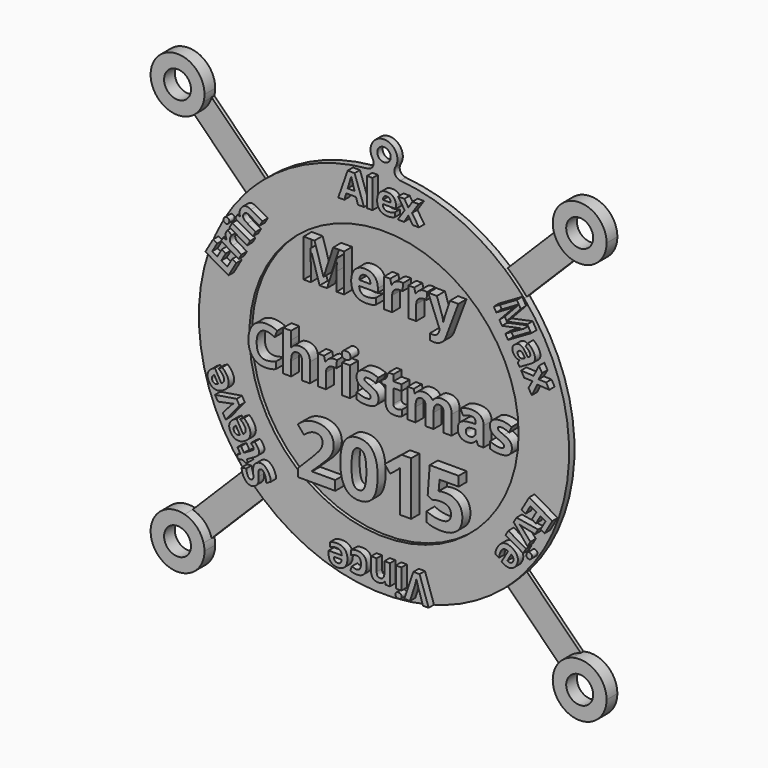
from build123d import *

# Parameters (mm, degrees)
F0_TEXT_SIZE   = 8.8194444444
F0_TEXT_SIZE_2 = 12.4976377996
F0_TEXT_SIZE_3 = 17.6388888889
F0_R           = 3.175
F1_DEPTH       = 3.175
F0_W           = 1.3132703993
F0_H           = 4.8148654514
F0_R_2         = 31.75
F0_H_2         = 6.7013997396
F0_R_3         = 1.5875
F2_DEPTH       = 1.5875
F0_W_2         = 1.8609763786
F0_H_3         = 6.8229291362
F3_DEPTH       = 0.79375


# Not quite as in the source:
# - Text() gives the source's letters only with a copy of the font that has no kerning and outlines rounded to 1/6400 em; it was checked with that copy


with BuildPart() as f1:
    # F0 (on Front) → F1 (new body)
    with BuildSketch(Plane.XZ):
        with Locations((-141.9037809198, 49.1509219737)):
            Text('Alex', F0_TEXT_SIZE, font='Open Sans', font_style=FontStyle.BOLD, text_align=(TextAlign.LEFT, TextAlign.BOTTOM))
        with Locations(Location((-105.6248470292, 39.1384926437), (0, 0, -60))):
            Text('Max', F0_TEXT_SIZE, font='Open Sans', font_style=FontStyle.BOLD, text_align=(TextAlign.LEFT, TextAlign.BOTTOM))
        with Locations((-151.1950764155, 29.4723159239)):
            Text('Merry', F0_TEXT_SIZE_2, font='Open Sans', font_style=FontStyle.BOLD, text_align=(TextAlign.LEFT, TextAlign.BOTTOM))
        with Locations((-163.8118323253, 8.3953211816)):
            Text('Christmas', F0_TEXT_SIZE_2, font='Open Sans', font_style=FontStyle.BOLD, text_align=(TextAlign.LEFT, TextAlign.BOTTOM))
        with Locations((-152.1226231507, -11.9727610818)):
            Text('2015', F0_TEXT_SIZE_3, font='Open Sans', font_style=FontStyle.BOLD, text_align=(TextAlign.LEFT, TextAlign.BOTTOM))
        with Locations(Location((-96.4686062678, 2.251259165), (0, 0, -120))):
            Text('Evie', F0_TEXT_SIZE, font='Open Sans', font_style=FontStyle.BOLD, text_align=(TextAlign.LEFT, TextAlign.BOTTOM))
        with Locations(Location((-120.5896641663, -22.7901004033), (0, 0, 180))):
            Text('Vince', F0_TEXT_SIZE, font='Open Sans', font_style=FontStyle.BOLD, text_align=(TextAlign.LEFT, TextAlign.BOTTOM))
        with Locations(Location((-157.3302373781, -15.2184386463), (0, 0, 120))):
            Text('Steve', F0_TEXT_SIZE, font='Open Sans', font_style=FontStyle.BOLD, text_align=(TextAlign.LEFT, TextAlign.BOTTOM))
        with Locations(Location((-168.179658373, 23.8811367259), (0, 0, 60))):
            Text('Erin', F0_TEXT_SIZE, font='Open Sans', font_style=FontStyle.BOLD, text_align=(TextAlign.LEFT, TextAlign.BOTTOM))
        with BuildLine():
            ThreePointArc((-173.4468957823, 60.3091405564), (-184.8346894931, 64.1747756306), (-178.1533948459, 54.1755115595))
            ThreePointArc((-178.1533948459, 54.1755115595), (-175.3067677218, 55.8190124959), (-173.6632667854, 58.66563962))
            ThreePointArc((-173.6632667854, 58.66563962), (-173.5012209126, 59.4802992358), (-173.4468957823, 60.3091405564))
        make_face()
        with Locations((-179.7968957823, 60.3091405564)):
            Circle(F0_R, mode=Mode.SUBTRACT)
        with BuildLine():
            ThreePointArc((-91.1011852452, 58.66563962), (-89.4576843088, 55.8190124959), (-86.6110571847, 54.1755115595))
            ThreePointArc((-86.6110571847, 54.1755115595), (-81.101921174, 55.2713468456), (-78.6175562483, 60.3091405564))
            ThreePointArc((-78.6175562483, 60.3091405564), (-85.7963975688, 66.6048154262), (-91.1011852452, 58.66563962))
        make_face()
        with Locations((-84.9675562483, 60.3091405564)):
            Circle(F0_R, mode=Mode.SUBTRACT)
        with BuildLine():
            ThreePointArc((-91.1011852452, -32.8766980412), (-85.7963975688, -40.8158738473), (-78.6175562483, -34.5201989776))
            ThreePointArc((-78.6175562483, -34.5201989776), (-81.101921174, -29.4824052668), (-86.6110571847, -28.3865699807))
            ThreePointArc((-86.6110571847, -28.3865699807), (-89.4576843088, -30.0300709171), (-91.1011852452, -32.8766980412))
        make_face()
        with Locations((-84.9675562483, -34.5201989776)):
            Circle(F0_R, mode=Mode.SUBTRACT)
        with BuildLine():
            ThreePointArc((-173.4468957823, -34.5201989776), (-173.5012209126, -33.691357657), (-173.6632667854, -32.8766980412))
            ThreePointArc((-173.6632667854, -32.8766980412), (-175.3067677218, -30.0300709171), (-178.1533948459, -28.3865699807))
            ThreePointArc((-178.1533948459, -28.3865699807), (-184.8346894931, -38.3858340518), (-173.4468957823, -34.5201989776))
        make_face()
        with Locations((-179.7968957823, -34.5201989776)):
            Circle(F0_R, mode=Mode.SUBTRACT)
    extrude(amount=F1_DEPTH)

    # F0 (on Front) → F2 (join)
    with BuildSketch(Plane.XZ):
        with BuildLine():
            ThreePointArc((-103.8385821698, -20.1393011166), (-101.5117733921, -17.9759818337), (-99.3484541093, -15.6491730561))
            ThreePointArc((-99.3484541093, -15.6491730561), (-88.724813239, 12.8944707894), (-99.3484541093, 41.4381146349))
            ThreePointArc((-99.3484541093, 41.4381146349), (-101.5117733921, 43.7649234126), (-103.8385821698, 45.9282426954))
            ThreePointArc((-103.8385821698, 45.9282426954), (-115.3481914405, 53.0916268632), (-128.5003258245, 56.3789570026))
            ThreePointArc((-128.5003258245, 56.3789570026), (-129.7826953761, 57.2575093055), (-129.7001883899, 58.8097716586))
            ThreePointArc((-129.7001883899, 58.8097716586), (-132.3822260153, 63.6839771129), (-135.0642636406, 58.8097716586))
            ThreePointArc((-135.0642636406, 58.8097716586), (-134.9817566545, 57.2575093055), (-136.2641262061, 56.3789570026))
            ThreePointArc((-136.2641262061, 56.3789570026), (-149.41626059, 53.0916268632), (-160.9258698607, 45.9282426954))
            ThreePointArc((-160.9258698607, 45.9282426954), (-163.2526786384, 43.7649234126), (-165.4159979213, 41.4381146349))
            ThreePointArc((-165.4159979213, 41.4381146349), (-176.0396387915, 12.8944707894), (-165.4159979213, -15.6491730561))
            ThreePointArc((-165.4159979213, -15.6491730561), (-163.2526786384, -17.9759818337), (-160.9258698607, -20.1393011166))
            ThreePointArc((-160.9258698607, -20.1393011166), (-132.3822260153, -30.7629419868), (-103.8385821698, -20.1393011166))
        make_face()
        with BuildLine():
            add(Edge.make_bspline(
                [(-161.8359432741, -12.9912476833), (-161.6326098639, -12.495937991), (-161.0991528745, -12.1879464546)],
                knots=[0, 0, 0, 1, 1, 1], degree=2))
            add(Edge.make_bspline(
                [(-161.0991528745, -12.1879464546), (-160.3604283186, -11.7614436334), (-159.6280174769, -12.0474751906)],
                knots=[0, 0, 0, 1, 1, 1], degree=2))
            add(Edge.make_bspline(
                [(-159.6280174769, -12.0474751906), (-158.8956066353, -12.3335067477), (-158.3492144912, -13.2798857022)],
                knots=[0, 0, 0, 1, 1, 1], degree=2))
            add(Edge.make_bspline(
                [(-158.3492144912, -13.2798857022), (-157.844852512, -14.1534662755), (-157.7870066185, -15.0143353854)],
                knots=[0, 0, 0, 1, 1, 1], degree=2))
            Line((-157.7870066185, -15.0143353854), (-158.8610810939, -15.6344525729))
            add(Edge.make_bspline(
                [(-158.8610810939, -15.6344525729), (-158.9323707875, -14.9404673891), (-159.0529544571, -14.50009993)],
                knots=[0, 0, 0, 1, 1, 1], degree=2))
            add(Edge.make_bspline(
                [(-159.0529544571, -14.50009993), (-159.1735381267, -14.059732471), (-159.3568172066, -13.7422837927)],
                knots=[0, 0, 0, 1, 1, 1], degree=2))
            add(Edge.make_bspline(
                [(-159.3568172066, -13.7422837927), (-159.5759252795, -13.3627774781), (-159.8384030897, -13.2430158561)],
                knots=[0, 0, 0, 1, 1, 1], degree=2))
            add(Edge.make_bspline(
                [(-159.8384030897, -13.2430158561), (-160.1008809, -13.1232542342), (-160.3884941762, -13.2893078366)],
                knots=[0, 0, 0, 1, 1, 1], degree=2))
            add(Edge.make_bspline(
                [(-160.3884941762, -13.2893078366), (-160.5484119314, -13.3816363956), (-160.6220441879, -13.5434896071)],
                knots=[0, 0, 0, 1, 1, 1], degree=2))
            add(Edge.make_bspline(
                [(-160.6220441879, -13.5434896071), (-160.6956764444, -13.7053428186), (-160.7105888179, -13.9454752017)],
                knots=[0, 0, 0, 1, 1, 1], degree=2))
            add(Edge.make_bspline(
                [(-160.7105888179, -13.9454752017), (-160.7255011913, -14.1856075847), (-160.6717072807, -14.8658256419)],
                knots=[0, 0, 0, 1, 1, 1], degree=2))
            add(Edge.make_bspline(
                [(-160.6717072807, -14.8658256419), (-160.6188002665, -15.5004103271), (-160.6904590768, -15.8751434532)],
                knots=[0, 0, 0, 1, 1, 1], degree=2))
            add(Edge.make_bspline(
                [(-160.6904590768, -15.8751434532), (-160.7621178871, -16.2498765794), (-160.9636037762, -16.5651071923)],
                knots=[0, 0, 0, 1, 1, 1], degree=2))
            add(Edge.make_bspline(
                [(-160.9636037762, -16.5651071923), (-161.1650896652, -16.8803378052), (-161.5481762281, -17.1015129354)],
                knots=[0, 0, 0, 1, 1, 1], degree=2))
            add(Edge.make_bspline(
                [(-161.5481762281, -17.1015129354), (-162.272579791, -17.5197475274), (-162.9692853129, -17.2679986342)],
                knots=[0, 0, 0, 1, 1, 1], degree=2))
            add(Edge.make_bspline(
                [(-162.9692853129, -17.2679986342), (-163.6659908349, -17.0162497409), (-164.1655296804, -16.1510230802)],
                knots=[0, 0, 0, 1, 1, 1], degree=2))
            add(Edge.make_bspline(
                [(-164.1655296804, -16.1510230802), (-164.410820479, -15.7261669543), (-164.5334712059, -15.2822192471)],
                knots=[0, 0, 0, 1, 1, 1], degree=2))
            add(Edge.make_bspline(
                [(-164.5334712059, -15.2822192471), (-164.6561219328, -14.8382715398), (-164.7167530134, -14.3115757404)],
                knots=[0, 0, 0, 1, 1, 1], degree=2))
            Line((-164.7167530134, -14.3115757404), (-163.6019433279, -14.1644011592))
            add(Edge.make_bspline(
                [(-163.6019433279, -14.1644011592), (-163.5287747508, -14.7045443104), (-163.4351074436, -15.0307673908)],
                knots=[0, 0, 0, 1, 1, 1], degree=2))
            add(Edge.make_bspline(
                [(-163.4351074436, -15.0307673908), (-163.3414401363, -15.3569904711), (-163.1822767249, -15.6326695864)],
                knots=[0, 0, 0, 1, 1, 1], degree=2))
            add(Edge.make_bspline(
                [(-163.1822767249, -15.6326695864), (-162.9927964731, -15.9608590094), (-162.7387534071, -16.0480967293)],
                knots=[0, 0, 0, 1, 1, 1], degree=2))
            add(Edge.make_bspline(
                [(-162.7387534071, -16.0480967293), (-162.4847103411, -16.1353344492), (-162.2388666279, -15.9933965152)],
                knots=[0, 0, 0, 1, 1, 1], degree=2))
            add(Edge.make_bspline(
                [(-162.2388666279, -15.9933965152), (-162.0861093691, -15.9052020707), (-162.0131347694, -15.7683924899)],
                knots=[0, 0, 0, 1, 1, 1], degree=2))
            add(Edge.make_bspline(
                [(-162.0131347694, -15.7683924899), (-161.9401601697, -15.6315829092), (-161.9231741113, -15.4157128267)],
                knots=[0, 0, 0, 1, 1, 1], degree=2))
            add(Edge.make_bspline(
                [(-161.9231741113, -15.4157128267), (-161.906188053, -15.1998427442), (-161.9639941807, -14.4630659482)],
                knots=[0, 0, 0, 1, 1, 1], degree=2))
            add(Edge.make_bspline(
                [(-161.9639941807, -14.4630659482), (-162.0392766843, -13.4865573756), (-161.8359432741, -12.9912476833)],
                knots=[0, 0, 0, 1, 1, 1], degree=2))
        make_face(mode=Mode.SUBTRACT)
        with BuildLine():
            add(Edge.make_bspline(
                [(-143.1674419441, -22.7873443269), (-142.7760790969, -22.703283997), (-142.2110834371, -22.703283997)],
                knots=[0, 0, 0, 1, 1, 1], degree=2))
            add(Edge.make_bspline(
                [(-142.2110834371, -22.703283997), (-141.0493972392, -22.703283997), (-140.3948290969, -23.3454497956)],
                knots=[0, 0, 0, 1, 1, 1], degree=2))
            add(Edge.make_bspline(
                [(-140.3948290969, -23.3454497956), (-139.7402609545, -23.9876155942), (-139.7402609545, -25.1630821741)],
                knots=[0, 0, 0, 1, 1, 1], degree=2))
            add(Edge.make_bspline(
                [(-139.7402609545, -25.1630821741), (-139.7402609545, -26.3729997088), (-140.3452197219, -27.0337690231)],
                knots=[0, 0, 0, 1, 1, 1], degree=2))
            add(Edge.make_bspline(
                [(-140.3452197219, -27.0337690231), (-140.9501784892, -27.6945383373), (-142.0181580899, -27.6945383373)],
                knots=[0, 0, 0, 1, 1, 1], degree=2))
            add(Edge.make_bspline(
                [(-142.0181580899, -27.6945383373), (-143.0379063538, -27.6945383373), (-143.606347109, -27.1136952383)],
                knots=[0, 0, 0, 1, 1, 1], degree=2))
            add(Edge.make_bspline(
                [(-143.606347109, -27.1136952383), (-144.1747878642, -26.5328521394), (-144.1747878642, -25.5075917227)],
                knots=[0, 0, 0, 1, 1, 1], degree=2))
            Line((-144.1747878642, -25.5075917227), (-144.1747878642, -24.8695600387))
            Line((-144.1747878642, -24.8695600387), (-141.0700678121, -24.8695600387))
            add(Edge.make_bspline(
                [(-141.0700678121, -24.8695600387), (-141.0921164233, -24.3100765317), (-141.402175017, -23.9958838234)],
                knots=[0, 0, 0, 1, 1, 1], degree=2))
            add(Edge.make_bspline(
                [(-141.402175017, -23.9958838234), (-141.7122336108, -23.6816911151), (-142.2717171177, -23.6816911151)],
                knots=[0, 0, 0, 1, 1, 1], degree=2))
            add(Edge.make_bspline(
                [(-142.2717171177, -23.6816911151), (-142.7071771871, -23.6816911151), (-143.0944059198, -23.7719526168)],
                knots=[0, 0, 0, 1, 1, 1], degree=2))
            add(Edge.make_bspline(
                [(-143.0944059198, -23.7719526168), (-143.4816346524, -23.8622141186), (-143.9033143399, -24.0606516186)],
                knots=[0, 0, 0, 1, 1, 1], degree=2))
            Line((-143.9033143399, -24.0606516186), (-143.9033143399, -23.0436594311))
            add(Edge.make_bspline(
                [(-143.9033143399, -23.0436594311), (-143.5588047913, -22.8714046567), (-143.1674419441, -22.7873443269)],
                knots=[0, 0, 0, 1, 1, 1], degree=2))
        make_face(mode=Mode.SUBTRACT)
        with BuildLine():
            add(Edge.make_bspline(
                [(-138.2726502774, -22.781143155), (-137.9474332635, -22.703283997), (-137.4527175517, -22.703283997)],
                knots=[0, 0, 0, 1, 1, 1], degree=2))
            add(Edge.make_bspline(
                [(-137.4527175517, -22.703283997), (-135.2051372566, -22.703283997), (-135.2051372566, -25.1713504033)],
                knots=[0, 0, 0, 1, 1, 1], degree=2))
            add(Edge.make_bspline(
                [(-135.2051372566, -25.1713504033), (-135.2051372566, -26.3991824345), (-135.8162971958, -27.0468603859)],
                knots=[0, 0, 0, 1, 1, 1], degree=2))
            add(Edge.make_bspline(
                [(-135.8162971958, -27.0468603859), (-136.4274571351, -27.6945383373), (-137.5684727601, -27.6945383373)],
                knots=[0, 0, 0, 1, 1, 1], degree=2))
            add(Edge.make_bspline(
                [(-137.5684727601, -27.6945383373), (-138.4035639059, -27.6945383373), (-139.0677783156, -27.3679432852)],
                knots=[0, 0, 0, 1, 1, 1], degree=2))
            Line((-139.0677783156, -27.3679432852), (-138.6791715448, -26.3509510977))
            add(Edge.make_bspline(
                [(-138.6791715448, -26.3509510977), (-138.369112951, -26.4763525734), (-138.1024625604, -26.5562787887)],
                knots=[0, 0, 0, 1, 1, 1], degree=2))
            add(Edge.make_bspline(
                [(-138.1024625604, -26.5562787887), (-137.8358121698, -26.636205004), (-137.5684727601, -26.636205004)],
                knots=[0, 0, 0, 1, 1, 1], degree=2))
            add(Edge.make_bspline(
                [(-137.5684727601, -26.636205004), (-136.5432123434, -26.636205004), (-136.5432123434, -25.1796186324)],
                knots=[0, 0, 0, 1, 1, 1], degree=2))
            add(Edge.make_bspline(
                [(-136.5432123434, -25.1796186324), (-136.5432123434, -23.7671294831), (-137.5684727601, -23.7671294831)],
                knots=[0, 0, 0, 1, 1, 1], degree=2))
            add(Edge.make_bspline(
                [(-137.5684727601, -23.7671294831), (-137.9474332635, -23.7671294831), (-138.2705832201, -23.8684152904)],
                knots=[0, 0, 0, 1, 1, 1], degree=2))
            add(Edge.make_bspline(
                [(-138.2705832201, -23.8684152904), (-138.5937331767, -23.9697010977), (-138.9161941142, -24.1860530942)],
                knots=[0, 0, 0, 1, 1, 1], degree=2))
            Line((-138.9161941142, -24.1860530942), (-138.9161941142, -23.0615739276))
            add(Edge.make_bspline(
                [(-138.9161941142, -23.0615739276), (-138.5978672913, -22.859002313), (-138.2726502774, -22.781143155)],
                knots=[0, 0, 0, 1, 1, 1], degree=2))
        make_face(mode=Mode.SUBTRACT)
        with BuildLine():
            add(Edge.make_bspline(
                [(-161.8572639586, -9.5657232543), (-161.8200507756, -9.3628389683), (-161.9495863659, -9.1384767446)],
                knots=[0, 0, 0, 1, 1, 1], degree=2))
            add(Edge.make_bspline(
                [(-161.9495863659, -9.1384767446), (-162.1218411402, -8.8401227236), (-162.4930801773, -8.4975301759)],
                knots=[0, 0, 0, 1, 1, 1], degree=2))
            Line((-162.4930801773, -8.4975301759), (-161.646948174, -8.009015636))
            add(Edge.make_bspline(
                [(-161.646948174, -8.009015636), (-161.2107108019, -8.3236287062), (-160.8531098905, -8.9430116537)],
                knots=[0, 0, 0, 1, 1, 1], degree=2))
            add(Edge.make_bspline(
                [(-160.8531098905, -8.9430116537), (-160.4589909669, -9.6256456536), (-160.6246509387, -10.1365982801)],
                knots=[0, 0, 0, 1, 1, 1], degree=2))
            add(Edge.make_bspline(
                [(-160.6246509387, -10.1365982801), (-160.7903109106, -10.6475509067), (-161.480105407, -11.0458039449)],
                knots=[0, 0, 0, 1, 1, 1], degree=2))
            Line((-161.480105407, -11.0458039449), (-163.4898180921, -12.2061121046))
            Line((-163.4898180921, -12.2061121046), (-163.1756253838, -12.7503098388))
            Line((-163.1756253838, -12.7503098388), (-163.6565720655, -13.027984535))
            Line((-163.6565720655, -13.027984535), (-164.3990068223, -12.621238183))
            Line((-164.3990068223, -12.621238183), (-165.4692281439, -12.8015448537))
            Line((-165.4692281439, -12.8015448537), (-165.8888407741, -12.0747544587))
            Line((-165.8888407741, -12.0747544587), (-165.0009392078, -11.5621242504))
            Line((-165.0009392078, -11.5621242504), (-165.6747998848, -10.3949633204))
            Line((-165.6747998848, -10.3949633204), (-164.8203139689, -9.9016256468))
            Line((-164.8203139689, -9.9016256468), (-164.1464532918, -11.0687865767))
            Line((-164.1464532918, -11.0687865767), (-162.1367406067, -9.908478417))
            add(Edge.make_bspline(
                [(-162.1367406067, -9.908478417), (-161.8944771417, -9.7686075403), (-161.8572639586, -9.5657232543)],
                knots=[0, 0, 0, 1, 1, 1], degree=2))
        make_face(mode=Mode.SUBTRACT)
        with BuildLine():
            Line((-165.8692510499, -0.4284331201), (-165.1953903729, -1.59559405))
            Line((-165.1953903729, -1.59559405), (-168.4481017512, -5.5914635832))
            Line((-168.4481017512, -5.5914635832), (-169.1350537911, -4.4016277477))
            Line((-169.1350537911, -4.4016277477), (-167.2240502589, -2.2242348686))
            add(Edge.make_bspline(
                [(-167.2240502589, -2.2242348686), (-166.8501091181, -1.8301230485), (-166.4679094517, -1.5633145463)],
                knots=[0, 0, 0, 1, 1, 1], degree=2))
            Line((-166.4679094517, -1.5633145463), (-166.4803117955, -1.5418330568))
            add(Edge.make_bspline(
                [(-166.4803117955, -1.5418330568), (-166.8493609262, -1.7294441286), (-167.4307559881, -1.8662100435)],
                knots=[0, 0, 0, 1, 1, 1], degree=2))
            Line((-167.4307559881, -1.8662100435), (-170.2698682442, -2.4360714577))
            Line((-170.2698682442, -2.4360714577), (-170.9568202841, -1.2462356222))
            Line((-170.9568202841, -1.2462356222), (-165.8692510499, -0.4284331201))
        make_face(mode=Mode.SUBTRACT)
        with BuildLine():
            add(Edge.make_bspline(
                [(-163.5827659105, -4.3832293996), (-163.3142861058, -4.6801294025), (-163.0317882759, -5.1694299968)],
                knots=[0, 0, 0, 1, 1, 1], degree=2))
            add(Edge.make_bspline(
                [(-163.0317882759, -5.1694299968), (-162.4509451769, -6.1754797554), (-162.6797930008, -7.0634352945)],
                knots=[0, 0, 0, 1, 1, 1], degree=2))
            add(Edge.make_bspline(
                [(-162.6797930008, -7.0634352945), (-162.9086408247, -7.9513908336), (-163.9266247441, -8.5391241236)],
                knots=[0, 0, 0, 1, 1, 1], degree=2))
            add(Edge.make_bspline(
                [(-163.9266247441, -8.5391241236), (-164.9744440657, -9.1440828909), (-165.8491664615, -8.9505578873)],
                knots=[0, 0, 0, 1, 1, 1], degree=2))
            add(Edge.make_bspline(
                [(-165.8491664615, -8.9505578873), (-166.7238888574, -8.7570328836), (-167.2578786577, -7.8321354187)],
                knots=[0, 0, 0, 1, 1, 1], degree=2))
            add(Edge.make_bspline(
                [(-167.2578786577, -7.8321354187), (-167.7677527897, -6.9490075167), (-167.548948288, -6.1663018327)],
                knots=[0, 0, 0, 1, 1, 1], degree=2))
            add(Edge.make_bspline(
                [(-167.548948288, -6.1663018327), (-167.3301437862, -5.3835961486), (-166.4422422199, -4.8709659403)],
                knots=[0, 0, 0, 1, 1, 1], degree=2))
            Line((-166.4422422199, -4.8709659403), (-165.8896905731, -4.5519500983))
            Line((-165.8896905731, -4.5519500983), (-164.3373305471, -7.240716535))
            add(Edge.make_bspline(
                [(-164.3373305471, -7.240716535), (-163.8638279226, -6.9418801242), (-163.7467583524, -6.5162651512)],
                knots=[0, 0, 0, 1, 1, 1], degree=2))
            add(Edge.make_bspline(
                [(-163.7467583524, -6.5162651512), (-163.6296887822, -6.0906501782), (-163.9094305357, -5.6061232482)],
                knots=[0, 0, 0, 1, 1, 1], degree=2))
            add(Edge.make_bspline(
                [(-163.9094305357, -5.6061232482), (-164.1271605704, -5.2290037657), (-164.3989436902, -4.938784597)],
                knots=[0, 0, 0, 1, 1, 1], degree=2))
            add(Edge.make_bspline(
                [(-164.3989436902, -4.938784597), (-164.67072681, -4.6485654283), (-165.0534185698, -4.3825988567)],
                knots=[0, 0, 0, 1, 1, 1], degree=2))
            Line((-165.0534185698, -4.3825988567), (-164.1726775, -3.874102763))
            add(Edge.make_bspline(
                [(-164.1726775, -3.874102763), (-163.8512457152, -4.0863293968), (-163.5827659105, -4.3832293996)],
                knots=[0, 0, 0, 1, 1, 1], degree=2))
        make_face(mode=Mode.SUBTRACT)
        with BuildLine():
            add(Edge.make_bspline(
                [(-168.6966656501, 4.4743047742), (-168.4281858453, 4.1774047713), (-168.1456880155, 3.6881041769)],
                knots=[0, 0, 0, 1, 1, 1], degree=2))
            add(Edge.make_bspline(
                [(-168.1456880155, 3.6881041769), (-167.5648449165, 2.6820544183), (-167.7936927404, 1.7940988792)],
                knots=[0, 0, 0, 1, 1, 1], degree=2))
            add(Edge.make_bspline(
                [(-167.7936927404, 1.7940988792), (-168.0225405642, 0.9061433401), (-169.0405244837, 0.3184100502)],
                knots=[0, 0, 0, 1, 1, 1], degree=2))
            add(Edge.make_bspline(
                [(-169.0405244837, 0.3184100502), (-170.0883438052, -0.2865487172), (-170.9630662011, -0.0930237135)],
                knots=[0, 0, 0, 1, 1, 1], degree=2))
            add(Edge.make_bspline(
                [(-170.9630662011, -0.0930237135), (-171.8377885969, 0.1005012902), (-172.3717783973, 1.0253987551)],
                knots=[0, 0, 0, 1, 1, 1], degree=2))
            add(Edge.make_bspline(
                [(-172.3717783973, 1.0253987551), (-172.8816525292, 1.9085266571), (-172.6628480275, 2.6912323411)],
                knots=[0, 0, 0, 1, 1, 1], degree=2))
            add(Edge.make_bspline(
                [(-172.6628480275, 2.6912323411), (-172.4440435258, 3.4739380251), (-171.5561419595, 3.9865682335)],
                knots=[0, 0, 0, 1, 1, 1], degree=2))
            Line((-171.5561419595, 3.9865682335), (-171.0035903127, 4.3055840755))
            Line((-171.0035903127, 4.3055840755), (-169.4512302867, 1.6168176387))
            add(Edge.make_bspline(
                [(-169.4512302867, 1.6168176387), (-168.9777276622, 1.9156540496), (-168.860658092, 2.3412690226)],
                knots=[0, 0, 0, 1, 1, 1], degree=2))
            add(Edge.make_bspline(
                [(-168.860658092, 2.3412690226), (-168.7435885218, 2.7668839956), (-169.0233302752, 3.2514109256)],
                knots=[0, 0, 0, 1, 1, 1], degree=2))
            add(Edge.make_bspline(
                [(-169.0233302752, 3.2514109256), (-169.24106031, 3.6285304081), (-169.5128434298, 3.9187495767)],
                knots=[0, 0, 0, 1, 1, 1], degree=2))
            add(Edge.make_bspline(
                [(-169.5128434298, 3.9187495767), (-169.7846265496, 4.2089687454), (-170.1673183094, 4.4749353171)],
                knots=[0, 0, 0, 1, 1, 1], degree=2))
            Line((-170.1673183094, 4.4749353171), (-169.2865772396, 4.9834314108))
            add(Edge.make_bspline(
                [(-169.2865772396, 4.9834314108), (-168.9651454548, 4.771204777), (-168.6966656501, 4.4743047742)],
                knots=[0, 0, 0, 1, 1, 1], degree=2))
        make_face(mode=Mode.SUBTRACT)
        with BuildLine():
            add(Edge.make_bspline(
                [(-127.6686463712, -28.2030344311), (-126.9534445483, -28.2030344311), (-126.9534445483, -28.8493343442)],
                knots=[0, 0, 0, 1, 1, 1], degree=2))
            add(Edge.make_bspline(
                [(-126.9534445483, -28.8493343442), (-126.9534445483, -29.4915001429), (-127.6686463712, -29.4915001429)],
                knots=[0, 0, 0, 1, 1, 1], degree=2))
            add(Edge.make_bspline(
                [(-127.6686463712, -29.4915001429), (-128.3838481941, -29.4915001429), (-128.3838481941, -28.8493343442)],
                knots=[0, 0, 0, 1, 1, 1], degree=2))
            add(Edge.make_bspline(
                [(-128.3838481941, -28.8493343442), (-128.3838481941, -28.5434098651), (-128.2053922479, -28.3732221481)],
                knots=[0, 0, 0, 1, 1, 1], degree=2))
            add(Edge.make_bspline(
                [(-128.2053922479, -28.3732221481), (-128.0269363017, -28.2030344311), (-127.6686463712, -28.2030344311)],
                knots=[0, 0, 0, 1, 1, 1], degree=2))
        make_face(mode=Mode.SUBTRACT)
        with BuildLine():
            Line((-134.1454258851, -25.9292714102), (-134.1454258851, -22.7901004033))
            Line((-134.1454258851, -22.7901004033), (-132.8321554858, -22.7901004033))
            Line((-132.8321554858, -22.7901004033), (-132.8321554858, -25.6026763581))
            add(Edge.make_bspline(
                [(-132.8321554858, -25.6026763581), (-132.8321554858, -26.1235747956), (-132.6468093486, -26.3840240144)],
                knots=[0, 0, 0, 1, 1, 1], degree=2))
            add(Edge.make_bspline(
                [(-132.6468093486, -26.3840240144), (-132.4614632115, -26.6444732331), (-132.0563199823, -26.6444732331)],
                knots=[0, 0, 0, 1, 1, 1], degree=2))
            add(Edge.make_bspline(
                [(-132.0563199823, -26.6444732331), (-131.5051047045, -26.6444732331), (-131.2598139059, -26.2765370352)],
                knots=[0, 0, 0, 1, 1, 1], degree=2))
            add(Edge.make_bspline(
                [(-131.2598139059, -26.2765370352), (-131.0145231073, -25.9086008373), (-131.0145231073, -25.0555951949)],
                knots=[0, 0, 0, 1, 1, 1], degree=2))
            Line((-131.0145231073, -25.0555951949), (-131.0145231073, -22.7901004033))
            Line((-131.0145231073, -22.7901004033), (-129.701252708, -22.7901004033))
            Line((-129.701252708, -22.7901004033), (-129.701252708, -27.6049658547))
            Line((-129.701252708, -27.6049658547), (-130.7044645135, -27.6049658547))
            Line((-130.7044645135, -27.6049658547), (-130.8808534024, -26.9889827817))
            Line((-130.8808534024, -26.9889827817), (-130.9538894267, -26.9889827817))
            add(Edge.make_bspline(
                [(-130.9538894267, -26.9889827817), (-131.1743755378, -27.3376264449), (-131.5595372132, -27.5160823911)],
                knots=[0, 0, 0, 1, 1, 1], degree=2))
            add(Edge.make_bspline(
                [(-131.5595372132, -27.5160823911), (-131.9446988885, -27.6945383373), (-132.4352804858, -27.6945383373)],
                knots=[0, 0, 0, 1, 1, 1], degree=2))
            add(Edge.make_bspline(
                [(-132.4352804858, -27.6945383373), (-133.2758837844, -27.6945383373), (-133.7106548347, -27.2404747522)],
                knots=[0, 0, 0, 1, 1, 1], degree=2))
            add(Edge.make_bspline(
                [(-133.7106548347, -27.2404747522), (-134.1454258851, -26.7864111672), (-134.1454258851, -25.9292714102)],
                knots=[0, 0, 0, 1, 1, 1], degree=2))
        make_face(mode=Mode.SUBTRACT)
        with Locations((-127.6665793139, -25.197533129)):
            Rectangle(F0_W, F0_H, mode=Mode.SUBTRACT)
        with BuildLine():
            Line((-123.7812006246, -25.339471063), (-124.9732036628, -29.0863569137))
            Line((-124.9732036628, -29.0863569137), (-126.320925017, -29.0863569137))
            Line((-126.320925017, -29.0863569137), (-124.180831701, -22.7901004033))
            Line((-124.180831701, -22.7901004033), (-122.7256233677, -22.7901004033))
            Line((-122.7256233677, -22.7901004033), (-120.5896641663, -29.0863569137))
            Line((-120.5896641663, -29.0863569137), (-121.9373855205, -29.0863569137))
            Line((-121.9373855205, -29.0863569137), (-123.1224983677, -25.339471063))
            add(Edge.make_bspline(
                [(-123.1224983677, -25.339471063), (-123.2203390795, -25.0073638581), (-123.3264480205, -24.5663916359)],
                knots=[0, 0, 0, 1, 1, 1], degree=2))
            add(Edge.make_bspline(
                [(-123.3264480205, -24.5663916359), (-123.4325569615, -24.1254194137), (-123.457361649, -23.9531646394)],
                knots=[0, 0, 0, 1, 1, 1], degree=2))
            add(Edge.make_bspline(
                [(-123.457361649, -23.9531646394), (-123.5055929858, -24.3486616012), (-123.7812006246, -25.339471063)],
                knots=[0, 0, 0, 1, 1, 1], degree=2))
        make_face(mode=Mode.SUBTRACT)
        with BuildLine():
            add(Edge.make_bspline(
                [(-104.706838369, -12.0122652462), (-104.5839553265, -11.6313049134), (-104.3014574967, -11.1420043191)],
                knots=[0, 0, 0, 1, 1, 1], degree=2))
            add(Edge.make_bspline(
                [(-104.3014574967, -11.1420043191), (-103.7206143977, -10.1359545605), (-102.8371984315, -9.89016482)],
                knots=[0, 0, 0, 1, 1, 1], degree=2))
            add(Edge.make_bspline(
                [(-102.8371984315, -9.89016482), (-101.9537824653, -9.6443750795), (-100.9357985458, -10.2321083694)],
                knots=[0, 0, 0, 1, 1, 1], degree=2))
            add(Edge.make_bspline(
                [(-100.9357985458, -10.2321083694), (-99.8879792243, -10.8370671368), (-99.6182155958, -11.6913614547)],
                knots=[0, 0, 0, 1, 1, 1], degree=2))
            add(Edge.make_bspline(
                [(-99.6182155958, -11.6913614547), (-99.3484519673, -12.5456557726), (-99.8824417676, -13.4705532375)],
                knots=[0, 0, 0, 1, 1, 1], degree=2))
            add(Edge.make_bspline(
                [(-99.8824417676, -13.4705532375), (-100.3923158996, -14.3536811395), (-101.1795611565, -14.5555437246)],
                knots=[0, 0, 0, 1, 1, 1], degree=2))
            add(Edge.make_bspline(
                [(-101.1795611565, -14.5555437246), (-101.9668064134, -14.7574063096), (-102.8547079797, -14.2447761013)],
                knots=[0, 0, 0, 1, 1, 1], degree=2))
            Line((-102.8547079797, -14.2447761013), (-103.4072596265, -13.9257602593))
            Line((-103.4072596265, -13.9257602593), (-101.8548996005, -11.2369938226))
            add(Edge.make_bspline(
                [(-101.8548996005, -11.2369938226), (-102.350450836, -10.9763467264), (-102.777579, -11.0877689911)],
                knots=[0, 0, 0, 1, 1, 1], degree=2))
            add(Edge.make_bspline(
                [(-102.777579, -11.0877689911), (-103.204707164, -11.1991912558), (-103.4844489175, -11.6837181858)],
                knots=[0, 0, 0, 1, 1, 1], degree=2))
            add(Edge.make_bspline(
                [(-103.4844489175, -11.6837181858), (-103.7021789522, -12.0608376683), (-103.817624565, -12.4413183387)],
                knots=[0, 0, 0, 1, 1, 1], degree=2))
            add(Edge.make_bspline(
                [(-103.817624565, -12.4413183387), (-103.9330701778, -12.8217990091), (-103.9720581055, -13.2862030807)],
                knots=[0, 0, 0, 1, 1, 1], degree=2))
            Line((-103.9720581055, -13.2862030807), (-104.8527991754, -12.777706987))
            add(Edge.make_bspline(
                [(-104.8527991754, -12.777706987), (-104.8297214115, -12.3932255789), (-104.706838369, -12.0122652462)],
                knots=[0, 0, 0, 1, 1, 1], degree=2))
        make_face(mode=Mode.SUBTRACT)
        Polygon((-98.2781181967, -10.5126383357), (-102.4479139935, -8.10520561), (-101.7912787938, -6.9678800821), (-97.6214829971, -9.3753128078), align=None, mode=Mode.SUBTRACT)
        with BuildLine():
            add(Edge.make_bspline(
                [(-97.4328915452, -10.2447999841), (-97.0752906337, -9.6254170366), (-96.5155784905, -9.9485669932)],
                knots=[0, 0, 0, 1, 1, 1], degree=2))
            add(Edge.make_bspline(
                [(-96.5155784905, -9.9485669932), (-95.9594465954, -10.2696498925), (-96.3170475069, -10.88903284)],
                knots=[0, 0, 0, 1, 1, 1], degree=2))
            add(Edge.make_bspline(
                [(-96.3170475069, -10.88903284), (-96.6746484183, -11.5084157875), (-97.2307803134, -11.1873328882)],
                knots=[0, 0, 0, 1, 1, 1], degree=2))
            add(Edge.make_bspline(
                [(-97.2307803134, -11.1873328882), (-97.495718684, -11.0343706486), (-97.5538775972, -10.7947294072)],
                knots=[0, 0, 0, 1, 1, 1], degree=2))
            add(Edge.make_bspline(
                [(-97.5538775972, -10.7947294072), (-97.6120365105, -10.5550881659), (-97.4328915452, -10.2447999841)],
                knots=[0, 0, 0, 1, 1, 1], degree=2))
        make_face(mode=Mode.SUBTRACT)
        with BuildLine():
            Line((-100.5289958077, -4.7815418167), (-99.8551351306, -3.6143808867))
            Line((-99.8551351306, -3.6143808867), (-94.7682549155, -4.4333768049))
            Line((-94.7682549155, -4.4333768049), (-95.4552069554, -5.6232126405))
            Line((-95.4552069554, -5.6232126405), (-98.2963862688, -5.0569314744))
            add(Edge.make_bspline(
                [(-98.2963862688, -5.0569314744), (-98.8246676874, -4.9301448571), (-99.2468304615, -4.7325544877)],
                knots=[0, 0, 0, 1, 1, 1], degree=2))
            Line((-99.2468304615, -4.7325544877), (-99.2592328052, -4.7540359772))
            add(Edge.make_bspline(
                [(-99.2592328052, -4.7540359772), (-98.9122322856, -4.9798363637), (-98.503091998, -5.4149562996)],
                knots=[0, 0, 0, 1, 1, 1], degree=2))
            Line((-98.503091998, -5.4149562996), (-96.5900214086, -7.5887689304))
            Line((-96.5900214086, -7.5887689304), (-97.2769734485, -8.778604766))
            Line((-97.2769734485, -8.778604766), (-100.5289958077, -4.7815418167))
        make_face(mode=Mode.SUBTRACT)
        Polygon((-97.7228686264, -2.1260480774), (-98.6776014935, -1.5748327996), (-96.8647922487, 1.5650449168), (-91.4120741619, -1.5830833384), (-93.2248834067, -4.7229610548), (-94.1724557772, -4.1758798916), (-93.0273060376, -2.1924223604), (-94.2243023696, -1.5013362058), (-95.290214913, -3.3475508874), (-96.2377872836, -2.8004697242), (-95.1718747402, -0.9542550426), (-96.5777188868, -0.1425905461), align=None, mode=Mode.SUBTRACT)
        Polygon((-166.9253960143, 28.2584439682), (-165.9706631473, 27.7072286904), (-167.7834723921, 24.567350974), (-173.2361904789, 27.7154792292), (-171.4233812341, 30.8553569457), (-170.4758088636, 30.3082757825), (-171.6209586031, 28.3248182512), (-170.4239622711, 27.6337320967), (-169.3580497277, 29.4799467783), (-168.4104773572, 28.9328656151), (-169.4763899006, 27.0866509335), (-168.0705457539, 26.274986437), align=None, mode=Mode.SUBTRACT)
        with BuildLine():
            add(Edge.make_bspline(
                [(-168.4697117825, 32.69290964), (-168.4934161891, 33.1465681151), (-168.2694849825, 33.5344283424)],
                knots=[0, 0, 0, 1, 1, 1], degree=2))
            add(Edge.make_bspline(
                [(-168.2694849825, 33.5344283424), (-168.1358152777, 33.7659510626), (-168.0142051829, 33.8994157866)],
                knots=[0, 0, 0, 1, 1, 1], degree=2))
            Line((-168.0142051829, 33.8994157866), (-166.9980939951, 33.1981957748))
            add(Edge.make_bspline(
                [(-166.9980939951, 33.1981957748), (-167.1150161089, 33.0811191011), (-167.22870426, 32.8842054473)],
                knots=[0, 0, 0, 1, 1, 1], degree=2))
            add(Edge.make_bspline(
                [(-167.22870426, 32.8842054473), (-167.5428969683, 32.340007713), (-167.4387407664, 31.8741116334)],
                knots=[0, 0, 0, 1, 1, 1], degree=2))
            add(Edge.make_bspline(
                [(-167.4387407664, 31.8741116334), (-167.3345845646, 31.4082155537), (-166.8309629772, 31.1174494947)],
                knots=[0, 0, 0, 1, 1, 1], degree=2))
            Line((-166.8309629772, 31.1174494947), (-164.7090691803, 29.8923735398))
            Line((-164.7090691803, 29.8923735398), (-165.3657043799, 28.755048012))
            Line((-165.3657043799, 28.755048012), (-169.5355001767, 31.1624807377))
            Line((-169.5355001767, 31.1624807377), (-169.0380283885, 32.0241271502))
            Line((-169.0380283885, 32.0241271502), (-168.2391480385, 31.7872555888))
            Line((-168.2391480385, 31.7872555888), (-168.20745316, 31.8421527287))
            add(Edge.make_bspline(
                [(-168.20745316, 31.8421527287), (-168.4460073758, 32.2392511649), (-168.4697117825, 32.69290964)],
                knots=[0, 0, 0, 1, 1, 1], degree=2))
        make_face(mode=Mode.SUBTRACT)
        with BuildLine():
            add(Edge.make_bspline(
                [(-167.721802132, 35.5000350534), (-168.0794030435, 34.8806521059), (-168.6391151868, 35.2038020625)],
                knots=[0, 0, 0, 1, 1, 1], degree=2))
            add(Edge.make_bspline(
                [(-168.6391151868, 35.2038020625), (-169.1952470818, 35.5248849618), (-168.8376461703, 36.1442679093)],
                knots=[0, 0, 0, 1, 1, 1], degree=2))
            add(Edge.make_bspline(
                [(-168.8376461703, 36.1442679093), (-168.4800452589, 36.7636508568), (-167.9239133638, 36.4425679575)],
                knots=[0, 0, 0, 1, 1, 1], degree=2))
            add(Edge.make_bspline(
                [(-167.9239133638, 36.4425679575), (-167.6589749932, 36.2896057179), (-167.60081608, 36.0499644765)],
                knots=[0, 0, 0, 1, 1, 1], degree=2))
            add(Edge.make_bspline(
                [(-167.60081608, 36.0499644765), (-167.5426571667, 35.8103232352), (-167.721802132, 35.5000350534)],
                knots=[0, 0, 0, 1, 1, 1], degree=2))
        make_face(mode=Mode.SUBTRACT)
        Polygon((-166.8765754805, 35.767873405), (-162.7067796838, 33.3604406793), (-163.3634148834, 32.2231151514), (-167.5332106801, 34.6305478771), align=None, mode=Mode.SUBTRACT)
        with BuildLine():
            Line((-162.5142758368, 39.9722091367), (-159.795673998, 38.4026236332))
            Line((-159.795673998, 38.4026236332), (-160.4523091977, 37.2652981054))
            Line((-160.4523091977, 37.2652981054), (-162.8880714246, 38.6715860828))
            add(Edge.make_bspline(
                [(-162.8880714246, 38.6715860828), (-163.3391827043, 38.9320353016), (-163.6574114127, 38.9017454477)],
                knots=[0, 0, 0, 1, 1, 1], degree=2))
            add(Edge.make_bspline(
                [(-163.6574114127, 38.9017454477), (-163.9756401211, 38.8714555938), (-164.1782117357, 38.5205912652)],
                knots=[0, 0, 0, 1, 1, 1], degree=2))
            add(Edge.make_bspline(
                [(-164.1782117357, 38.5205912652), (-164.4538193746, 38.0432248317), (-164.2578226795, 37.6468286698)],
                knots=[0, 0, 0, 1, 1, 1], degree=2))
            add(Edge.make_bspline(
                [(-164.2578226795, 37.6468286698), (-164.0618259845, 37.2504325079), (-163.3231014286, 36.8239296867)],
                knots=[0, 0, 0, 1, 1, 1], degree=2))
            Line((-163.3231014286, 36.8239296867), (-161.3611253869, 35.6911822909))
            Line((-161.3611253869, 35.6911822909), (-162.0177605865, 34.5538567631))
            Line((-162.0177605865, 34.5538567631), (-166.1875563832, 36.9612894888))
            Line((-166.1875563832, 36.9612894888), (-165.6859504805, 37.8300963977))
            Line((-165.6859504805, 37.8300963977), (-165.0642990466, 37.67486212))
            Line((-165.0642990466, 37.67486212), (-165.0277810344, 37.7381131724))
            add(Edge.make_bspline(
                [(-165.0277810344, 37.7381131724), (-165.2194722481, 38.1033815774), (-165.1814387932, 38.526169346)],
                knots=[0, 0, 0, 1, 1, 1], degree=2))
            add(Edge.make_bspline(
                [(-165.1814387932, 38.526169346), (-165.1434053384, 38.9489571145), (-164.8981145398, 39.3738132403)],
                knots=[0, 0, 0, 1, 1, 1], degree=2))
            add(Edge.make_bspline(
                [(-164.8981145398, 39.3738132403), (-164.4778128905, 40.1017970514), (-163.8671967657, 40.2512880333)],
                knots=[0, 0, 0, 1, 1, 1], degree=2))
            add(Edge.make_bspline(
                [(-163.8671967657, 40.2512880333), (-163.2565806409, 40.4007790152), (-162.5142758368, 39.9722091367)],
                knots=[0, 0, 0, 1, 1, 1], degree=2))
        make_face(mode=Mode.SUBTRACT)
        with Locations((-132.3822260153, 12.8944707894)):
            Circle(F0_R_2, mode=Mode.SUBTRACT)
        Polygon((-135.8183642531, 49.1509219737), (-137.2570361281, 49.1509219737), (-137.7131667705, 50.6502275292), (-140.0089784024, 50.6502275292), (-140.4651090448, 49.1509219737), (-141.9037809198, 49.1509219737), (-139.6810053121, 55.4733612098), (-138.0494080899, 55.4733612098), align=None, mode=Mode.SUBTRACT)
        with Locations((-134.4727099562, 52.5016218434)):
            Rectangle(F0_W, F0_H_2, mode=Mode.SUBTRACT)
        with Locations((-132.3822260153, 60.5089771129)):
            Circle(F0_R_3, mode=Mode.SUBTRACT)
        Polygon((-98.7821983746, 27.2866775157), (-95.836656451, 27.1016895259), (-94.5710614321, 29.6225052764), (-93.826231788, 28.3324224898), (-94.6873489413, 26.7564081298), (-92.8877877776, 26.7069897837), (-92.1422691144, 25.4157135811), (-94.9671143503, 25.5955984282), (-96.2755468989, 22.9450298029), (-97.0231326194, 24.2398862538), (-96.1003535845, 25.9406095187), (-98.0366797114, 25.9954013131), align=None, mode=Mode.SUBTRACT)
        with BuildLine():
            Line((-99.1356651715, 27.8988999667), (-99.5938628712, 28.6925216624))
            Line((-99.5938628712, 28.6925216624), (-99.1544587644, 29.2405877091))
            Line((-99.1544587644, 29.2405877091), (-99.1716842418, 29.2704231112))
            add(Edge.make_bspline(
                [(-99.1716842418, 29.2704231112), (-99.6986538985, 29.3480701848), (-100.0145801581, 29.5714315423)],
                knots=[0, 0, 0, 1, 1, 1], degree=2))
            add(Edge.make_bspline(
                [(-100.0145801581, 29.5714315423), (-100.3305064178, 29.7947928997), (-100.6123152285, 30.282900078)],
                knots=[0, 0, 0, 1, 1, 1], degree=2))
            add(Edge.make_bspline(
                [(-100.6123152285, 30.282900078), (-100.9588918344, 30.8831883681), (-100.8143145214, 31.4265231163)],
                knots=[0, 0, 0, 1, 1, 1], degree=2))
            add(Edge.make_bspline(
                [(-100.8143145214, 31.4265231163), (-100.6697372084, 31.9698578645), (-100.0360332679, 32.3357270051)],
                knots=[0, 0, 0, 1, 1, 1], degree=2))
            add(Edge.make_bspline(
                [(-100.0360332679, 32.3357270051), (-99.3724939253, 32.7188216232), (-98.7894036504, 32.4364838083)],
                knots=[0, 0, 0, 1, 1, 1], degree=2))
            add(Edge.make_bspline(
                [(-98.7894036504, 32.4364838083), (-98.2063133755, 32.1541459934), (-97.6327067529, 31.2378003184)],
                knots=[0, 0, 0, 1, 1, 1], degree=2))
            Line((-97.6327067529, 31.2378003184), (-97.1917972553, 30.5264881184))
            Line((-97.1917972553, 30.5264881184), (-97.0092045945, 30.6319080403))
            add(Edge.make_bspline(
                [(-97.0092045945, 30.6319080403), (-96.375500654, 30.9977771809), (-96.7503270429, 31.6469955305)],
                knots=[0, 0, 0, 1, 1, 1], degree=2))
            add(Edge.make_bspline(
                [(-96.7503270429, 31.6469955305), (-97.0390260446, 32.1470368696), (-97.7309451228, 32.6481885414)],
                knots=[0, 0, 0, 1, 1, 1], degree=2))
            Line((-97.7309451228, 32.6481885414), (-97.1794261805, 33.4678429064))
            add(Edge.make_bspline(
                [(-97.1794261805, 33.4678429064), (-96.3868281824, 32.9659430426), (-95.881088165, 32.0899756371)],
                knots=[0, 0, 0, 1, 1, 1], degree=2))
            add(Edge.make_bspline(
                [(-95.881088165, 32.0899756371), (-95.3967077397, 31.2510041302), (-95.5041076079, 30.5922887455)],
                knots=[0, 0, 0, 1, 1, 1], degree=2))
            add(Edge.make_bspline(
                [(-95.5041076079, 30.5922887455), (-95.6115074761, 29.9335733608), (-96.3573925285, 29.502936425)],
                knots=[0, 0, 0, 1, 1, 1], degree=2))
            Line((-96.3573925285, 29.502936425), (-99.1356651715, 27.8988999667))
        make_face(mode=Mode.SUBTRACT)
        with BuildLine():
            Line((-103.2842491559, 35.0844582071), (-103.8960981142, 36.1442116895))
            Line((-103.8960981142, 36.1442116895), (-100.3768158769, 39.9264138261))
            Line((-100.3768158769, 39.9264138261), (-100.3961084116, 39.9598294764))
            add(Edge.make_bspline(
                [(-100.3961084116, 39.9598294764), (-101.6591710454, 39.1351266381), (-102.095961332, 38.8829456486)],
                knots=[0, 0, 0, 1, 1, 1], degree=2))
            Line((-102.095961332, 38.8829456486), (-104.6319705101, 37.418780067))
            Line((-104.6319705101, 37.418780067), (-105.2286610483, 38.4522783955))
            Line((-105.2286610483, 38.4522783955), (-99.7759429615, 41.6004066507))
            Line((-99.7759429615, 41.6004066507), (-98.8671267723, 40.0262908362))
            Line((-98.8671267723, 40.0262908362), (-102.2920929249, 36.328775324))
            Line((-102.2920929249, 36.328775324), (-102.279001562, 36.3061004184))
            Line((-102.279001562, 36.3061004184), (-97.3189008608, 37.344684896))
            Line((-97.3189008608, 37.344684896), (-96.4107736907, 35.7717624976))
            Line((-96.4107736907, 35.7717624976), (-101.8634917774, 32.6236342424))
            Line((-101.8634917774, 32.6236342424), (-102.4856760222, 33.701288966))
            Line((-102.4856760222, 33.701288966), (-99.904317033, 35.1916372733))
            add(Edge.make_bspline(
                [(-99.904317033, 35.1916372733), (-99.7217243722, 35.2970571952), (-99.47959606, 35.4288939342)],
                knots=[0, 0, 0, 1, 1, 1], degree=2))
            add(Edge.make_bspline(
                [(-99.47959606, 35.4288939342), (-99.2374677477, 35.5607306732), (-98.1832493769, 36.1105087399)],
                knots=[0, 0, 0, 1, 1, 1], degree=2))
            Line((-98.1832493769, 36.1105087399), (-98.2025419116, 36.1439243903))
            Line((-98.2025419116, 36.1439243903), (-103.2842491559, 35.0844582071))
        make_face(mode=Mode.SUBTRACT)
        with BuildLine():
            add(Edge.make_bspline(
                [(-129.3029996698, 49.1481658973), (-129.694362517, 49.0641055674), (-130.2593581767, 49.0641055674)],
                knots=[0, 0, 0, 1, 1, 1], degree=2))
            add(Edge.make_bspline(
                [(-130.2593581767, 49.0641055674), (-131.4210443746, 49.0641055674), (-132.075612517, 49.706271366)],
                knots=[0, 0, 0, 1, 1, 1], degree=2))
            add(Edge.make_bspline(
                [(-132.075612517, 49.706271366), (-132.7301806594, 50.3484371646), (-132.7301806594, 51.5239037445)],
                knots=[0, 0, 0, 1, 1, 1], degree=2))
            add(Edge.make_bspline(
                [(-132.7301806594, 51.5239037445), (-132.7301806594, 52.7338212792), (-132.125221892, 53.3945905934)],
                knots=[0, 0, 0, 1, 1, 1], degree=2))
            add(Edge.make_bspline(
                [(-132.125221892, 53.3945905934), (-131.5202631246, 54.0553599077), (-130.452283524, 54.0553599077)],
                knots=[0, 0, 0, 1, 1, 1], degree=2))
            add(Edge.make_bspline(
                [(-130.452283524, 54.0553599077), (-129.4325352601, 54.0553599077), (-128.8640945049, 53.4745168087)],
                knots=[0, 0, 0, 1, 1, 1], degree=2))
            add(Edge.make_bspline(
                [(-128.8640945049, 53.4745168087), (-128.2956537496, 52.8936737098), (-128.2956537496, 51.8684132931)],
                knots=[0, 0, 0, 1, 1, 1], degree=2))
            Line((-128.2956537496, 51.8684132931), (-128.2956537496, 51.2303816091))
            Line((-128.2956537496, 51.2303816091), (-131.4003738017, 51.2303816091))
            add(Edge.make_bspline(
                [(-131.4003738017, 51.2303816091), (-131.3783251906, 50.6708981021), (-131.0682665969, 50.3567053938)],
                knots=[0, 0, 0, 1, 1, 1], degree=2))
            add(Edge.make_bspline(
                [(-131.0682665969, 50.3567053938), (-130.7582080031, 50.0425126855), (-130.1987244962, 50.0425126855)],
                knots=[0, 0, 0, 1, 1, 1], degree=2))
            add(Edge.make_bspline(
                [(-130.1987244962, 50.0425126855), (-129.7632644267, 50.0425126855), (-129.3760356941, 50.1327741872)],
                knots=[0, 0, 0, 1, 1, 1], degree=2))
            add(Edge.make_bspline(
                [(-129.3760356941, 50.1327741872), (-128.9888069615, 50.2230356889), (-128.567127274, 50.4214731889)],
                knots=[0, 0, 0, 1, 1, 1], degree=2))
            Line((-128.567127274, 50.4214731889), (-128.567127274, 49.4044810014))
            add(Edge.make_bspline(
                [(-128.567127274, 49.4044810014), (-128.9116368226, 49.2322262271), (-129.3029996698, 49.1481658973)],
                knots=[0, 0, 0, 1, 1, 1], degree=2))
        make_face(mode=Mode.SUBTRACT)
        Polygon((-127.8739740621, 49.1509219737), (-126.2409988017, 51.6093421125), (-127.7912917705, 53.965787425), (-126.3016324823, 53.965787425), (-125.3673225865, 52.4320309146), (-124.4247444615, 53.965787425), (-122.9337071351, 53.965787425), (-124.5019146003, 51.6093421125), (-122.8606711108, 49.1509219737), (-124.3558425517, 49.1509219737), (-125.3673225865, 50.8004336924), (-126.3829367358, 49.1509219737), align=None, mode=Mode.SUBTRACT)
        with BuildLine():
            add(Edge.make_bspline(
                [(-166.5551589652, -6.6514951713), (-166.661649454, -6.9962149009), (-166.4528766675, -7.3578199743)],
                knots=[0, 0, 0, 1, 1, 1], degree=2))
            add(Edge.make_bspline(
                [(-166.4528766675, -7.3578199743), (-166.244103881, -7.7194250477), (-165.8964567082, -7.7924009474)],
                knots=[0, 0, 0, 1, 1, 1], degree=2))
            add(Edge.make_bspline(
                [(-165.8964567082, -7.7924009474), (-165.5488095354, -7.8653768471), (-165.1103081804, -7.6519885079)],
                knots=[0, 0, 0, 1, 1, 1], degree=2))
            Line((-165.1103081804, -7.6519885079), (-166.0322157325, -6.0551977878))
            add(Edge.make_bspline(
                [(-166.0322157325, -6.0551977878), (-166.4486684764, -6.3067754417), (-166.5551589652, -6.6514951713)],
                knots=[0, 0, 0, 1, 1, 1], degree=2))
        make_face()
        with BuildLine():
            add(Edge.make_bspline(
                [(-171.6690587048, 2.2060390025), (-171.7755491935, 1.8613192729), (-171.5667764071, 1.4997141995)],
                knots=[0, 0, 0, 1, 1, 1], degree=2))
            add(Edge.make_bspline(
                [(-171.5667764071, 1.4997141995), (-171.3580036206, 1.1381091261), (-171.0103564478, 1.0651332264)],
                knots=[0, 0, 0, 1, 1, 1], degree=2))
            add(Edge.make_bspline(
                [(-171.0103564478, 1.0651332264), (-170.662709275, 0.9921573266), (-170.22420792, 1.2055456659)],
                knots=[0, 0, 0, 1, 1, 1], degree=2))
            Line((-170.22420792, 1.2055456659), (-171.1461154721, 2.8023363859))
            add(Edge.make_bspline(
                [(-171.1461154721, 2.8023363859), (-171.562568216, 2.550758732), (-171.6690587048, 2.2060390025)],
                knots=[0, 0, 0, 1, 1, 1], degree=2))
        make_face()
        with BuildLine():
            add(Edge.make_bspline(
                [(-142.6892626906, -26.4956451081), (-142.443971892, -26.7602284415), (-142.0264263191, -26.7602284415)],
                knots=[0, 0, 0, 1, 1, 1], degree=2))
            add(Edge.make_bspline(
                [(-142.0264263191, -26.7602284415), (-141.6088807462, -26.7602284415), (-141.3718581767, -26.4956451081)],
                knots=[0, 0, 0, 1, 1, 1], degree=2))
            add(Edge.make_bspline(
                [(-141.3718581767, -26.4956451081), (-141.1348356073, -26.2310617748), (-141.1003846524, -25.7446142922)],
                knots=[0, 0, 0, 1, 1, 1], degree=2))
            Line((-141.1003846524, -25.7446142922), (-142.9441997566, -25.7446142922))
            add(Edge.make_bspline(
                [(-142.9441997566, -25.7446142922), (-142.9345534892, -26.2310617748), (-142.6892626906, -26.4956451081)],
                knots=[0, 0, 0, 1, 1, 1], degree=2))
        make_face()
        with BuildLine():
            add(Edge.make_bspline(
                [(-101.2562660608, -13.4523002557), (-100.9044847735, -13.3721638595), (-100.695711987, -13.0105587861)],
                knots=[0, 0, 0, 1, 1, 1], degree=2))
            add(Edge.make_bspline(
                [(-100.695711987, -13.0105587861), (-100.4869392005, -12.6489537127), (-100.5975638039, -12.3113944796)],
                knots=[0, 0, 0, 1, 1, 1], degree=2))
            add(Edge.make_bspline(
                [(-100.5975638039, -12.3113944796), (-100.7081884073, -11.9738352465), (-101.1122388074, -11.7007761031)],
                knots=[0, 0, 0, 1, 1, 1], degree=2))
            Line((-101.1122388074, -11.7007761031), (-102.0341463595, -13.2975668232))
            add(Edge.make_bspline(
                [(-102.0341463595, -13.2975668232), (-101.6080473482, -13.532436652), (-101.2562660608, -13.4523002557)],
                knots=[0, 0, 0, 1, 1, 1], degree=2))
        make_face()
        with BuildLine():
            Line((-98.19904043, 29.9449560003), (-97.8553365979, 30.1433935003))
            Line((-97.8553365979, 30.1433935003), (-98.1250990538, 30.574806787))
            add(Edge.make_bspline(
                [(-98.1250990538, 30.574806787), (-98.4260519913, 31.0629996487), (-98.7300175795, 31.2105229878)],
                knots=[0, 0, 0, 1, 1, 1], degree=2))
            add(Edge.make_bspline(
                [(-98.7300175795, 31.2105229878), (-99.0339831678, 31.358046327), (-99.3693330873, 31.1644319606)],
                knots=[0, 0, 0, 1, 1, 1], degree=2))
            add(Edge.make_bspline(
                [(-99.3693330873, 31.1644319606), (-99.8514731852, 30.8860682454), (-99.5331463623, 30.3347100147)],
                knots=[0, 0, 0, 1, 1, 1], degree=2))
            add(Edge.make_bspline(
                [(-99.5331463623, 30.3347100147), (-99.304392022, 29.9384958748), (-98.9396792592, 29.8332054298)],
                knots=[0, 0, 0, 1, 1, 1], degree=2))
            add(Edge.make_bspline(
                [(-98.9396792592, 29.8332054298), (-98.5749664964, 29.7279149847), (-98.19904043, 29.9449560003)],
                knots=[0, 0, 0, 1, 1, 1], degree=2))
        make_face()
        with BuildLine():
            add(Edge.make_bspline(
                [(-129.7811789233, 52.8564666785), (-130.0264697219, 53.1210500118), (-130.4440152948, 53.1210500118)],
                knots=[0, 0, 0, 1, 1, 1], degree=2))
            add(Edge.make_bspline(
                [(-130.4440152948, 53.1210500118), (-130.8615608677, 53.1210500118), (-131.0985834371, 52.8564666785)],
                knots=[0, 0, 0, 1, 1, 1], degree=2))
            add(Edge.make_bspline(
                [(-131.0985834371, 52.8564666785), (-131.3356060066, 52.5918833452), (-131.3700569615, 52.1054358625)],
                knots=[0, 0, 0, 1, 1, 1], degree=2))
            Line((-131.3700569615, 52.1054358625), (-129.5262418573, 52.1054358625))
            add(Edge.make_bspline(
                [(-129.5262418573, 52.1054358625), (-129.5358881246, 52.5918833452), (-129.7811789233, 52.8564666785)],
                knots=[0, 0, 0, 1, 1, 1], degree=2))
        make_face()
        with BuildLine():
            Line((-139.672737083, 51.7691945431), (-138.0328716316, 51.7691945431))
            add(Edge.make_bspline(
                [(-138.0328716316, 51.7691945431), (-138.6653911628, 53.8059349945), (-138.7453173781, 54.0732744042)],
                knots=[0, 0, 0, 1, 1, 1], degree=2))
            add(Edge.make_bspline(
                [(-138.7453173781, 54.0732744042), (-138.8252435934, 54.3406138139), (-138.8596945483, 54.4949540917)],
                knots=[0, 0, 0, 1, 1, 1], degree=2))
            add(Edge.make_bspline(
                [(-138.8596945483, 54.4949540917), (-139.0016324823, 53.9437388139), (-139.672737083, 51.7691945431)],
                knots=[0, 0, 0, 1, 1, 1], degree=2))
        make_face()
    extrude(amount=F2_DEPTH)

    # F0 (on Front) → F3 (join)
    with BuildSketch(Plane.XZ):
        with Locations((-132.3822260153, 12.8944707894)):
            Circle(F0_R_2)
        with BuildLine():
            add(Edge.make_bspline(
                [(-157.9047457091, 15.6937463809), (-158.4105094888, 15.8704707904), (-158.8986984654, 15.8704707904)],
                knots=[0, 0, 0, 1, 1, 1], degree=2))
            add(Edge.make_bspline(
                [(-158.8986984654, 15.8704707904), (-159.9668559461, 15.8704707904), (-160.5526827179, 15.067888113)],
                knots=[0, 0, 0, 1, 1, 1], degree=2))
            add(Edge.make_bspline(
                [(-160.5526827179, 15.067888113), (-161.1385094898, 14.2653054356), (-161.1385094898, 12.8319826004)],
                knots=[0, 0, 0, 1, 1, 1], degree=2))
            add(Edge.make_bspline(
                [(-161.1385094898, 12.8319826004), (-161.1385094898, 9.8481715758), (-158.8986984654, 9.8481715758)],
                knots=[0, 0, 0, 1, 1, 1], degree=2))
            add(Edge.make_bspline(
                [(-158.8986984654, 9.8481715758), (-157.9594228745, 9.8481715758), (-156.6237378347, 10.3168329932)],
                knots=[0, 0, 0, 1, 1, 1], degree=2))
            Line((-156.6237378347, 10.3168329932), (-156.6237378347, 8.7311951974))
            add(Edge.make_bspline(
                [(-156.6237378347, 8.7311951974), (-157.7211866539, 8.2722975595), (-159.0763992528, 8.2722975595)],
                knots=[0, 0, 0, 1, 1, 1], degree=2))
            add(Edge.make_bspline(
                [(-159.0763992528, 8.2722975595), (-161.0232968913, 8.2722975595), (-162.0543520098, 9.4537148827)],
                knots=[0, 0, 0, 1, 1, 1], degree=2))
            add(Edge.make_bspline(
                [(-162.0543520098, 9.4537148827), (-163.0854071282, 10.635132206), (-163.0854071282, 12.8436991359)],
                knots=[0, 0, 0, 1, 1, 1], degree=2))
            add(Edge.make_bspline(
                [(-163.0854071282, 12.8436991359), (-163.0854071282, 14.236014097), (-162.5786669706, 15.2826912627)],
                knots=[0, 0, 0, 1, 1, 1], degree=2))
            add(Edge.make_bspline(
                [(-162.5786669706, 15.2826912627), (-162.0719268129, 16.3293684284), (-161.1228874425, 16.8868802396)],
                knots=[0, 0, 0, 1, 1, 1], degree=2))
            add(Edge.make_bspline(
                [(-161.1228874425, 16.8868802396), (-160.1738480721, 17.4443920508), (-158.8986984654, 17.4443920508)],
                knots=[0, 0, 0, 1, 1, 1], degree=2))
            add(Edge.make_bspline(
                [(-158.8986984654, 17.4443920508), (-157.6001157878, 17.4443920508), (-156.2878638188, 16.8175574049)],
                knots=[0, 0, 0, 1, 1, 1], degree=2))
            Line((-156.2878638188, 16.8175574049), (-156.8971236615, 15.2787857509))
            add(Edge.make_bspline(
                [(-156.8971236615, 15.2787857509), (-157.3989819294, 15.5170219714), (-157.9047457091, 15.6937463809)],
                knots=[0, 0, 0, 1, 1, 1], degree=2))
        make_face(mode=Mode.SUBTRACT)
        with BuildLine():
            Line((-142.614159609, -9.7320709776), (-142.614159609, -11.9727610818))
            Line((-142.614159609, -11.9727610818), (-151.4170675951, -11.9727610818))
            Line((-151.4170675951, -11.9727610818), (-151.4170675951, -10.1206777485))
            Line((-151.4170675951, -10.1206777485), (-148.2558479771, -6.9263852137))
            add(Edge.make_bspline(
                [(-148.2558479771, -6.9263852137), (-146.8502490187, -5.4877133387), (-146.4203011021, -4.9323639464)],
                knots=[0, 0, 0, 1, 1, 1], degree=2))
            add(Edge.make_bspline(
                [(-146.4203011021, -4.9323639464), (-145.9903531854, -4.377014554), (-145.8001839146, -3.9029694151)],
                knots=[0, 0, 0, 1, 1, 1], degree=2))
            add(Edge.make_bspline(
                [(-145.8001839146, -3.9029694151), (-145.6100146437, -3.4289242762), (-145.6100146437, -2.9218062207)],
                knots=[0, 0, 0, 1, 1, 1], degree=2))
            add(Edge.make_bspline(
                [(-145.6100146437, -2.9218062207), (-145.6100146437, -2.1638852137), (-146.0289382549, -1.7931929394)],
                knots=[0, 0, 0, 1, 1, 1], degree=2))
            add(Edge.make_bspline(
                [(-146.0289382549, -1.7931929394), (-146.447861866, -1.4225006651), (-147.1451491924, -1.4225006651)],
                knots=[0, 0, 0, 1, 1, 1], degree=2))
            add(Edge.make_bspline(
                [(-147.1451491924, -1.4225006651), (-147.8755094354, -1.4225006651), (-148.5645285326, -1.7587419846)],
                knots=[0, 0, 0, 1, 1, 1], degree=2))
            add(Edge.make_bspline(
                [(-148.5645285326, -1.7587419846), (-149.2535476299, -2.094983304), (-150.0032004076, -2.7151004915)],
                knots=[0, 0, 0, 1, 1, 1], degree=2))
            Line((-150.0032004076, -2.7151004915), (-151.4501405118, -1.0008209776))
            add(Edge.make_bspline(
                [(-151.4501405118, -1.0008209776), (-150.5213427687, -0.2070709776), (-149.9094938104, 0.1195240745)],
                knots=[0, 0, 0, 1, 1, 1], degree=2))
            add(Edge.make_bspline(
                [(-149.9094938104, 0.1195240745), (-149.2976448521, 0.4461191265), (-148.5741748, 0.6225080154)],
                knots=[0, 0, 0, 1, 1, 1], degree=2))
            add(Edge.make_bspline(
                [(-148.5741748, 0.6225080154), (-147.8507047479, 0.7988969043), (-146.9549799215, 0.7988969043)],
                knots=[0, 0, 0, 1, 1, 1], degree=2))
            add(Edge.make_bspline(
                [(-146.9549799215, 0.7988969043), (-145.7753792271, 0.7988969043), (-144.8713861715, 0.3689489877)],
                knots=[0, 0, 0, 1, 1, 1], degree=2))
            add(Edge.make_bspline(
                [(-144.8713861715, 0.3689489877), (-143.967393116, -0.060998929), (-143.4671652514, -0.8368344325)],
                knots=[0, 0, 0, 1, 1, 1], degree=2))
            add(Edge.make_bspline(
                [(-143.4671652514, -0.8368344325), (-142.9669373868, -1.612669936), (-142.9669373868, -2.6103695887)],
                knots=[0, 0, 0, 1, 1, 1], degree=2))
            add(Edge.make_bspline(
                [(-142.9669373868, -2.6103695887), (-142.9669373868, -3.4812897276), (-143.272861866, -4.2433448491)],
                knots=[0, 0, 0, 1, 1, 1], degree=2))
            add(Edge.make_bspline(
                [(-143.272861866, -4.2433448491), (-143.5787863451, -5.0053999707), (-144.2209521437, -5.8060401616)],
                knots=[0, 0, 0, 1, 1, 1], degree=2))
            add(Edge.make_bspline(
                [(-144.2209521437, -5.8060401616), (-144.8631179424, -6.6066803526), (-146.4809347826, -8.0894494498)],
                knots=[0, 0, 0, 1, 1, 1], degree=2))
            Line((-146.4809347826, -8.0894494498), (-148.1015076993, -9.6135596929))
            Line((-148.1015076993, -9.6135596929), (-148.1015076993, -9.7320709776))
            Line((-148.1015076993, -9.7320709776), (-142.614159609, -9.7320709776))
        make_face(mode=Mode.SUBTRACT)
        with BuildLine():
            add(Edge.make_bspline(
                [(-133.7299473694, -0.8354563943), (-132.6151144701, -2.4891022276), (-132.6151144701, -5.6778826096)],
                knots=[0, 0, 0, 1, 1, 1], degree=2))
            add(Edge.make_bspline(
                [(-132.6151144701, -5.6778826096), (-132.6151144701, -8.9741499707), (-133.6954964146, -10.5602719325)],
                knots=[0, 0, 0, 1, 1, 1], degree=2))
            add(Edge.make_bspline(
                [(-133.6954964146, -10.5602719325), (-134.775878359, -12.1463938943), (-137.0248366924, -12.1463938943)],
                knots=[0, 0, 0, 1, 1, 1], degree=2))
            add(Edge.make_bspline(
                [(-137.0248366924, -12.1463938943), (-139.204893116, -12.1463938943), (-140.3114577861, -10.5092845193)],
                knots=[0, 0, 0, 1, 1, 1], degree=2))
            add(Edge.make_bspline(
                [(-140.3114577861, -10.5092845193), (-141.4180224562, -8.8721751443), (-141.4180224562, -5.6778826096)],
                knots=[0, 0, 0, 1, 1, 1], degree=2))
            add(Edge.make_bspline(
                [(-141.4180224562, -5.6778826096), (-141.4180224562, -2.343030179), (-140.3403965882, -0.76242037)],
                knots=[0, 0, 0, 1, 1, 1], degree=2))
            add(Edge.make_bspline(
                [(-140.3403965882, -0.76242037), (-139.2627707201, 0.818189439), (-137.0248366924, 0.818189439)],
                knots=[0, 0, 0, 1, 1, 1], degree=2))
            add(Edge.make_bspline(
                [(-137.0248366924, 0.818189439), (-134.8447802687, 0.818189439), (-133.7299473694, -0.8354563943)],
                knots=[0, 0, 0, 1, 1, 1], degree=2))
        make_face(mode=Mode.SUBTRACT)
        with BuildLine():
            add(Edge.make_bspline(
                [(-144.0255331059, 14.9946597665), (-143.4855960978, 15.3451794517), (-142.8509504283, 15.3451794517)],
                knots=[0, 0, 0, 1, 1, 1], degree=2))
            add(Edge.make_bspline(
                [(-142.8509504283, 15.3451794517), (-142.4721157825, 15.3451794517), (-142.2221630265, 15.2905022863)],
                knots=[0, 0, 0, 1, 1, 1], degree=2))
            Line((-142.2221630265, 15.2905022863), (-142.3627614518, 13.5466912621))
            add(Edge.make_bspline(
                [(-142.3627614518, 13.5466912621), (-142.5892811369, 13.6072266952), (-142.9114858614, 13.6072266952)],
                knots=[0, 0, 0, 1, 1, 1], degree=2))
            add(Edge.make_bspline(
                [(-142.9114858614, 13.6072266952), (-143.8019425547, 13.6072266952), (-144.2998953107, 13.1493054352)],
                knots=[0, 0, 0, 1, 1, 1], degree=2))
            add(Edge.make_bspline(
                [(-144.2998953107, 13.1493054352), (-144.7978480668, 12.6913841752), (-144.7978480668, 11.8673211828)],
                knots=[0, 0, 0, 1, 1, 1], degree=2))
            Line((-144.7978480668, 11.8673211828), (-144.7978480668, 8.3953211816))
            Line((-144.7978480668, 8.3953211816), (-146.6588244454, 8.3953211816))
            Line((-146.6588244454, 8.3953211816), (-146.6588244454, 15.2182503178))
            Line((-146.6588244454, 15.2182503178), (-145.2489346811, 15.2182503178))
            Line((-145.2489346811, 15.2182503178), (-144.9735960984, 14.0700298449))
            Line((-144.9735960984, 14.0700298449), (-144.8837693267, 14.0700298449))
            add(Edge.make_bspline(
                [(-144.8837693267, 14.0700298449), (-144.565470114, 14.6441400814), (-144.0255331059, 14.9946597665)],
                knots=[0, 0, 0, 1, 1, 1], degree=2))
        make_face(mode=Mode.SUBTRACT)
        with Locations((-140.0536275927, 11.8067857497)):
            Rectangle(F0_W_2, F0_H_3, mode=Mode.SUBTRACT)
        with BuildLine():
            add(Edge.make_bspline(
                [(-132.5872653854, 11.2941873243), (-132.409564598, 10.9280455919), (-132.409564598, 10.4222818122)],
                knots=[0, 0, 0, 1, 1, 1], degree=2))
            add(Edge.make_bspline(
                [(-132.409564598, 10.4222818122), (-132.409564598, 9.3716991347), (-133.1389189289, 8.8219983471)],
                knots=[0, 0, 0, 1, 1, 1], degree=2))
            add(Edge.make_bspline(
                [(-133.1389189289, 8.8219983471), (-133.8682732599, 8.2722975595), (-135.3211236541, 8.2722975595)],
                knots=[0, 0, 0, 1, 1, 1], degree=2))
            add(Edge.make_bspline(
                [(-135.3211236541, 8.2722975595), (-136.0651236543, 8.2722975595), (-136.5904149931, 8.3738408666)],
                knots=[0, 0, 0, 1, 1, 1], degree=2))
            add(Edge.make_bspline(
                [(-136.5904149931, 8.3738408666), (-137.1157063319, 8.4753841737), (-137.5726512139, 8.6706597643)],
                knots=[0, 0, 0, 1, 1, 1], degree=2))
            Line((-137.5726512139, 8.6706597643), (-137.5726512139, 10.2074786625))
            add(Edge.make_bspline(
                [(-137.5726512139, 10.2074786625), (-137.0551708988, 9.9633841742), (-136.404903182, 9.7983763002)],
                knots=[0, 0, 0, 1, 1, 1], degree=2))
            add(Edge.make_bspline(
                [(-136.404903182, 9.7983763002), (-135.7546354653, 9.6333684261), (-135.260588221, 9.6333684261)],
                knots=[0, 0, 0, 1, 1, 1], degree=2))
            add(Edge.make_bspline(
                [(-135.260588221, 9.6333684261), (-134.2471079057, 9.6333684261), (-134.2471079057, 10.2191951979)],
                knots=[0, 0, 0, 1, 1, 1], degree=2))
            add(Edge.make_bspline(
                [(-134.2471079057, 10.2191951979), (-134.2471079057, 10.4398566153), (-134.3818480632, 10.5775259067)],
                knots=[0, 0, 0, 1, 1, 1], degree=2))
            add(Edge.make_bspline(
                [(-134.3818480632, 10.5775259067), (-134.5165882207, 10.7151951981), (-134.8456275909, 10.8889904738)],
                knots=[0, 0, 0, 1, 1, 1], degree=2))
            add(Edge.make_bspline(
                [(-134.8456275909, 10.8889904738), (-135.1746669611, 11.0627857494), (-135.7233913708, 11.2932109463)],
                knots=[0, 0, 0, 1, 1, 1], degree=2))
            add(Edge.make_bspline(
                [(-135.7233913708, 11.2932109463), (-136.510352001, 11.6232266945), (-136.8803992452, 11.904423545)],
                knots=[0, 0, 0, 1, 1, 1], degree=2))
            add(Edge.make_bspline(
                [(-136.8803992452, 11.904423545), (-137.2504464894, 12.1856203955), (-137.4174071194, 12.548832994)],
                knots=[0, 0, 0, 1, 1, 1], degree=2))
            add(Edge.make_bspline(
                [(-137.4174071194, 12.548832994), (-137.5843677494, 12.9120455926), (-137.5843677494, 13.4412424431)],
                knots=[0, 0, 0, 1, 1, 1], degree=2))
            add(Edge.make_bspline(
                [(-137.5843677494, 13.4412424431), (-137.5843677494, 14.3512266954), (-136.8803992452, 14.8482030736)],
                knots=[0, 0, 0, 1, 1, 1], degree=2))
            add(Edge.make_bspline(
                [(-136.8803992452, 14.8482030736), (-136.176430741, 15.3451794517), (-134.8817535752, 15.3451794517)],
                knots=[0, 0, 0, 1, 1, 1], degree=2))
            add(Edge.make_bspline(
                [(-134.8817535752, 15.3451794517), (-133.6495645984, 15.3451794517), (-132.4837693224, 14.8081715775)],
                knots=[0, 0, 0, 1, 1, 1], degree=2))
            Line((-132.4837693224, 14.8081715775), (-133.0442102675, 13.4666282699))
            add(Edge.make_bspline(
                [(-133.0442102675, 13.4666282699), (-133.5577850708, 13.6853369314), (-134.0030134174, 13.8259353567)],
                knots=[0, 0, 0, 1, 1, 1], degree=2))
            add(Edge.make_bspline(
                [(-134.0030134174, 13.8259353567), (-134.448241764, 13.9665337819), (-134.9129976697, 13.9665337819)],
                knots=[0, 0, 0, 1, 1, 1], degree=2))
            add(Edge.make_bspline(
                [(-134.9129976697, 13.9665337819), (-135.7370606621, 13.9665337819), (-135.7370606621, 13.5213054353)],
                knots=[0, 0, 0, 1, 1, 1], degree=2))
            add(Edge.make_bspline(
                [(-135.7370606621, 13.5213054353), (-135.7370606621, 13.2713526793), (-135.4714858589, 13.0877936241)],
                knots=[0, 0, 0, 1, 1, 1], degree=2))
            add(Edge.make_bspline(
                [(-135.4714858589, 13.0877936241), (-135.2059110556, 12.9042345689), (-134.3076433388, 12.5449274822)],
                knots=[0, 0, 0, 1, 1, 1], degree=2))
            add(Edge.make_bspline(
                [(-134.3076433388, 12.5449274822), (-133.5089661731, 12.2207700018), (-133.136966173, 11.9405495292)],
                knots=[0, 0, 0, 1, 1, 1], degree=2))
            add(Edge.make_bspline(
                [(-133.136966173, 11.9405495292), (-132.7649661729, 11.6603290567), (-132.5872653854, 11.2941873243)],
                knots=[0, 0, 0, 1, 1, 1], degree=2))
        make_face(mode=Mode.SUBTRACT)
        with BuildLine():
            Line((-124.6996630812, 0.619751939), (-124.6996630812, -11.9727610818))
            Line((-124.6996630812, -11.9727610818), (-127.3620328729, -11.9727610818))
            Line((-127.3620328729, -11.9727610818), (-127.3620328729, -4.6856951096))
            Line((-127.3620328729, -4.6856951096), (-127.334472109, -3.4895579568))
            Line((-127.334472109, -3.4895579568), (-127.2931309632, -2.1804216721))
            add(Edge.make_bspline(
                [(-127.2931309632, -2.1804216721), (-127.9545892965, -2.8418800054), (-128.2136604771, -3.0485857346)],
                knots=[0, 0, 0, 1, 1, 1], degree=2))
            Line((-128.2136604771, -3.0485857346), (-129.6606005812, -4.2116499707))
            Line((-129.6606005812, -4.2116499707), (-130.9449321785, -2.6103695887))
            Line((-130.9449321785, -2.6103695887), (-126.887987734, 0.619751939))
            Line((-126.887987734, 0.619751939), (-124.6996630812, 0.619751939))
        make_face(mode=Mode.SUBTRACT)
        with BuildLine():
            add(Edge.make_bspline(
                [(-117.9307394701, -4.0490414637), (-117.4043288799, -3.9277741026), (-116.6298714146, -3.9277741026)],
                knots=[0, 0, 0, 1, 1, 1], degree=2))
            add(Edge.make_bspline(
                [(-116.6298714146, -3.9277741026), (-114.8053488451, -3.9277741026), (-113.7235888625, -4.9530345193)],
                knots=[0, 0, 0, 1, 1, 1], degree=2))
            add(Edge.make_bspline(
                [(-113.7235888625, -4.9530345193), (-112.6418288799, -5.978294936), (-112.6418288799, -7.7614763596)],
                knots=[0, 0, 0, 1, 1, 1], degree=2))
            add(Edge.make_bspline(
                [(-112.6418288799, -7.7614763596), (-112.6418288799, -9.8698747971), (-113.9426969354, -11.0081343457)],
                knots=[0, 0, 0, 1, 1, 1], degree=2))
            add(Edge.make_bspline(
                [(-113.9426969354, -11.0081343457), (-115.243564991, -12.1463938943), (-117.6634000604, -12.1463938943)],
                knots=[0, 0, 0, 1, 1, 1], degree=2))
            add(Edge.make_bspline(
                [(-117.6634000604, -12.1463938943), (-119.7662863451, -12.1463938943), (-121.0561300951, -11.4656430262)],
                knots=[0, 0, 0, 1, 1, 1], degree=2))
            Line((-121.0561300951, -11.4656430262), (-121.0561300951, -9.1643192415))
            add(Edge.make_bspline(
                [(-121.0561300951, -9.1643192415), (-120.3781353035, -9.5253652485), (-119.4727642097, -9.7541195887)],
                knots=[0, 0, 0, 1, 1, 1], degree=2))
            add(Edge.make_bspline(
                [(-119.4727642097, -9.7541195887), (-118.567393116, -9.982873929), (-117.759862734, -9.982873929)],
                knots=[0, 0, 0, 1, 1, 1], degree=2))
            add(Edge.make_bspline(
                [(-117.759862734, -9.982873929), (-115.3207351299, -9.982873929), (-115.3207351299, -7.9847185471)],
                knots=[0, 0, 0, 1, 1, 1], degree=2))
            add(Edge.make_bspline(
                [(-115.3207351299, -7.9847185471), (-115.3207351299, -6.0802697623), (-117.8453011021, -6.0802697623)],
                knots=[0, 0, 0, 1, 1, 1], degree=2))
            add(Edge.make_bspline(
                [(-117.8453011021, -6.0802697623), (-118.3000537062, -6.0802697623), (-118.851268984, -6.1712202832)],
                knots=[0, 0, 0, 1, 1, 1], degree=2))
            add(Edge.make_bspline(
                [(-118.851268984, -6.1712202832), (-119.4024842618, -6.262170804), (-119.7469938104, -6.3669017068)],
                knots=[0, 0, 0, 1, 1, 1], degree=2))
            Line((-119.7469938104, -6.3669017068), (-120.8080832201, -5.7963938943))
            Line((-120.8080832201, -5.7963938943), (-120.3340380812, 0.619751939))
            Line((-120.3340380812, 0.619751939), (-113.5044807896, 0.619751939))
            Line((-113.5044807896, 0.619751939), (-113.5044807896, -1.6374746235))
            Line((-113.5044807896, -1.6374746235), (-117.9996413799, -1.6374746235))
            Line((-117.9996413799, -1.6374746235), (-118.2311517965, -4.1096751443))
            Line((-118.2311517965, -4.1096751443), (-117.9307394701, -4.0490414637))
        make_face(mode=Mode.SUBTRACT)
        with BuildLine():
            add(Edge.make_bspline(
                [(-128.6739425494, 9.9458093711), (-128.4513283761, 9.7563920482), (-128.0842102658, 9.7563920482)],
                knots=[0, 0, 0, 1, 1, 1], degree=2))
            add(Edge.make_bspline(
                [(-128.0842102658, 9.7563920482), (-127.5960212892, 9.7563920482), (-126.912556722, 9.9692424419)],
                knots=[0, 0, 0, 1, 1, 1], degree=2))
            Line((-126.912556722, 9.9692424419), (-126.912556722, 8.5847385045))
            add(Edge.make_bspline(
                [(-126.912556722, 8.5847385045), (-127.6077378246, 8.2722975595), (-128.62121814, 8.2722975595)],
                knots=[0, 0, 0, 1, 1, 1], degree=2))
            add(Edge.make_bspline(
                [(-128.62121814, 8.2722975595), (-129.7381945183, 8.2722975595), (-130.2478638098, 8.8376203943)],
                knots=[0, 0, 0, 1, 1, 1], degree=2))
            add(Edge.make_bspline(
                [(-130.2478638098, 8.8376203943), (-130.7575331013, 9.4029432292), (-130.7575331013, 10.5316361429)],
                knots=[0, 0, 0, 1, 1, 1], degree=2))
            Line((-130.7575331013, 10.5316361429), (-130.7575331013, 13.8200770889))
            Line((-130.7575331013, 13.8200770889), (-131.6479897945, 13.8200770889))
            Line((-131.6479897945, 13.8200770889), (-131.6479897945, 14.6070377191))
            Line((-131.6479897945, 14.6070377191), (-130.6227929438, 15.2299668532))
            Line((-130.6227929438, 15.2299668532), (-130.0857850696, 16.671100712))
            Line((-130.0857850696, 16.671100712), (-128.8965567227, 16.671100712))
            Line((-128.8965567227, 16.671100712), (-128.8965567227, 15.2182503178))
            Line((-128.8965567227, 15.2182503178), (-126.9867614465, 15.2182503178))
            Line((-126.9867614465, 15.2182503178), (-126.9867614465, 13.8200770889))
            Line((-126.9867614465, 13.8200770889), (-128.8965567227, 13.8200770889))
            Line((-128.8965567227, 13.8200770889), (-128.8965567227, 10.5316361429))
            add(Edge.make_bspline(
                [(-128.8965567227, 10.5316361429), (-128.8965567227, 10.135226694), (-128.6739425494, 9.9458093711)],
                knots=[0, 0, 0, 1, 1, 1], degree=2))
        make_face(mode=Mode.SUBTRACT)
        with BuildLine():
            Line((-119.4256905777, 11.8185022851), (-119.4256905777, 8.3953211816))
            Line((-119.4256905777, 8.3953211816), (-121.2866669563, 8.3953211816))
            Line((-121.2866669563, 8.3953211816), (-121.2866669563, 12.3808959861))
            add(Edge.make_bspline(
                [(-121.2866669563, 12.3808959861), (-121.2866669563, 13.1190377186), (-121.5336905785, 13.4881085849)],
                knots=[0, 0, 0, 1, 1, 1], degree=2))
            add(Edge.make_bspline(
                [(-121.5336905785, 13.4881085849), (-121.7807142006, 13.8571794512), (-122.3118638071, 13.8571794512)],
                knots=[0, 0, 0, 1, 1, 1], degree=2))
            add(Edge.make_bspline(
                [(-122.3118638071, 13.8571794512), (-123.0265724687, 13.8571794512), (-123.3497535712, 13.3318881124)],
                knots=[0, 0, 0, 1, 1, 1], degree=2))
            add(Edge.make_bspline(
                [(-123.3497535712, 13.3318881124), (-123.6729346737, 12.8065967736), (-123.6729346737, 11.6056518913)],
                knots=[0, 0, 0, 1, 1, 1], degree=2))
            Line((-123.6729346737, 11.6056518913), (-123.6729346737, 8.3953211816))
            Line((-123.6729346737, 8.3953211816), (-125.5339110523, 8.3953211816))
            Line((-125.5339110523, 8.3953211816), (-125.5339110523, 15.2182503178))
            Line((-125.5339110523, 15.2182503178), (-124.1123047526, 15.2182503178))
            Line((-124.1123047526, 15.2182503178), (-123.8623519966, 14.3453684277))
            Line((-123.8623519966, 14.3453684277), (-123.7588559336, 14.3453684277))
            add(Edge.make_bspline(
                [(-123.7588559336, 14.3453684277), (-123.4835173508, 14.8159826011), (-122.9650606577, 15.0805810264)],
                knots=[0, 0, 0, 1, 1, 1], degree=2))
            add(Edge.make_bspline(
                [(-122.9650606577, 15.0805810264), (-122.4466039646, 15.3451794517), (-121.7748559329, 15.3451794517)],
                knots=[0, 0, 0, 1, 1, 1], degree=2))
            add(Edge.make_bspline(
                [(-121.7748559329, 15.3451794517), (-120.2438953024, 15.3451794517), (-119.6990764046, 14.3453684277)],
                knots=[0, 0, 0, 1, 1, 1], degree=2))
            Line((-119.6990764046, 14.3453684277), (-119.5350449085, 14.3453684277))
            add(Edge.make_bspline(
                [(-119.5350449085, 14.3453684277), (-119.2597063257, 14.8218408688), (-118.7266039633, 15.0835101602)],
                knots=[0, 0, 0, 1, 1, 1], degree=2))
            add(Edge.make_bspline(
                [(-118.7266039633, 15.0835101602), (-118.1935016009, 15.3451794517), (-117.5217535692, 15.3451794517)],
                knots=[0, 0, 0, 1, 1, 1], degree=2))
            add(Edge.make_bspline(
                [(-117.5217535692, 15.3451794517), (-116.3618165609, 15.3451794517), (-115.7672023875, 14.7505652782)],
                knots=[0, 0, 0, 1, 1, 1], degree=2))
            add(Edge.make_bspline(
                [(-115.7672023875, 14.7505652782), (-115.1725882141, 14.1559511048), (-115.1725882141, 12.8436991359)],
                knots=[0, 0, 0, 1, 1, 1], degree=2))
            Line((-115.1725882141, 12.8436991359), (-115.1725882141, 8.3953211816))
            Line((-115.1725882141, 8.3953211816), (-117.0394228604, 8.3953211816))
            Line((-117.0394228604, 8.3953211816), (-117.0394228604, 12.3808959861))
            add(Edge.make_bspline(
                [(-117.0394228604, 12.3808959861), (-117.0394228604, 13.1190377186), (-117.2864464825, 13.4881085849)],
                knots=[0, 0, 0, 1, 1, 1], degree=2))
            add(Edge.make_bspline(
                [(-117.2864464825, 13.4881085849), (-117.5334701046, 13.8571794512), (-118.0646197111, 13.8571794512)],
                knots=[0, 0, 0, 1, 1, 1], degree=2))
            add(Edge.make_bspline(
                [(-118.0646197111, 13.8571794512), (-118.7480842783, 13.8571794512), (-119.086887428, 13.3689904746)],
                knots=[0, 0, 0, 1, 1, 1], degree=2))
            add(Edge.make_bspline(
                [(-119.086887428, 13.3689904746), (-119.4256905777, 12.8808014981), (-119.4256905777, 11.8185022851)],
                knots=[0, 0, 0, 1, 1, 1], degree=2))
        make_face(mode=Mode.SUBTRACT)
        with BuildLine():
            Line((-107.6310449044, 8.3953211816), (-108.929627582, 8.3953211816))
            Line((-108.929627582, 8.3953211816), (-109.2908874246, 9.322880237))
            Line((-109.2908874246, 9.322880237), (-109.3397063223, 9.322880237))
            add(Edge.make_bspline(
                [(-109.3397063223, 9.322880237), (-109.8083677398, 8.7311951974), (-110.3063204958, 8.5017463784)],
                knots=[0, 0, 0, 1, 1, 1], degree=2))
            add(Edge.make_bspline(
                [(-110.3063204958, 8.5017463784), (-110.8042732519, 8.2722975595), (-111.6029504175, 8.2722975595)],
                knots=[0, 0, 0, 1, 1, 1], degree=2))
            add(Edge.make_bspline(
                [(-111.6029504175, 8.2722975595), (-112.5851866384, 8.2722975595), (-113.1495330952, 8.8346912605)],
                knots=[0, 0, 0, 1, 1, 1], degree=2))
            add(Edge.make_bspline(
                [(-113.1495330952, 8.8346912605), (-113.7138795521, 9.3970849614), (-113.7138795521, 10.4339983476)],
                knots=[0, 0, 0, 1, 1, 1], degree=2))
            add(Edge.make_bspline(
                [(-113.7138795521, 10.4339983476), (-113.7138795521, 11.5197306315), (-112.9542575046, 12.0352581907)],
                knots=[0, 0, 0, 1, 1, 1], degree=2))
            add(Edge.make_bspline(
                [(-112.9542575046, 12.0352581907), (-112.1946354571, 12.5507857499), (-110.6636748267, 12.6054629153)],
                knots=[0, 0, 0, 1, 1, 1], degree=2))
            Line((-110.6636748267, 12.6054629153), (-109.4783519916, 12.6425652775))
            Line((-109.4783519916, 12.6425652775), (-109.4783519916, 12.9413369312))
            add(Edge.make_bspline(
                [(-109.4783519916, 12.9413369312), (-109.4783519916, 13.9782503173), (-110.5406512046, 13.9782503173)],
                knots=[0, 0, 0, 1, 1, 1], degree=2))
            add(Edge.make_bspline(
                [(-110.5406512046, 13.9782503173), (-111.3588559293, 13.9782503173), (-112.4641157722, 13.4842030731)],
                knots=[0, 0, 0, 1, 1, 1], degree=2))
            Line((-112.4641157722, 13.4842030731), (-113.0792338826, 14.7417778767))
            add(Edge.make_bspline(
                [(-113.0792338826, 14.7417778767), (-111.9017220712, 15.358848743), (-110.468399236, 15.358848743)],
                knots=[0, 0, 0, 1, 1, 1], degree=2))
            add(Edge.make_bspline(
                [(-110.468399236, 15.358848743), (-109.095611834, 15.358848743), (-108.3633283692, 14.7603290578)],
                knots=[0, 0, 0, 1, 1, 1], degree=2))
            add(Edge.make_bspline(
                [(-108.3633283692, 14.7603290578), (-107.6310449044, 14.1618093725), (-107.6310449044, 12.9413369312)],
                knots=[0, 0, 0, 1, 1, 1], degree=2))
            Line((-107.6310449044, 12.9413369312), (-107.6310449044, 8.3953211816))
        make_face(mode=Mode.SUBTRACT)
        with BuildLine():
            add(Edge.make_bspline(
                [(-101.1303204927, 11.2941873243), (-100.9526197052, 10.9280455919), (-100.9526197052, 10.4222818122)],
                knots=[0, 0, 0, 1, 1, 1], degree=2))
            add(Edge.make_bspline(
                [(-100.9526197052, 10.4222818122), (-100.9526197052, 9.3716991347), (-101.6819740362, 8.8219983471)],
                knots=[0, 0, 0, 1, 1, 1], degree=2))
            add(Edge.make_bspline(
                [(-101.6819740362, 8.8219983471), (-102.4113283671, 8.2722975595), (-103.8641787613, 8.2722975595)],
                knots=[0, 0, 0, 1, 1, 1], degree=2))
            add(Edge.make_bspline(
                [(-103.8641787613, 8.2722975595), (-104.6081787616, 8.2722975595), (-105.1334701003, 8.3738408666)],
                knots=[0, 0, 0, 1, 1, 1], degree=2))
            add(Edge.make_bspline(
                [(-105.1334701003, 8.3738408666), (-105.6587614391, 8.4753841737), (-106.1157063212, 8.6706597643)],
                knots=[0, 0, 0, 1, 1, 1], degree=2))
            Line((-106.1157063212, 8.6706597643), (-106.1157063212, 10.2074786625))
            add(Edge.make_bspline(
                [(-106.1157063212, 10.2074786625), (-105.598226006, 9.9633841742), (-104.9479582893, 9.7983763002)],
                knots=[0, 0, 0, 1, 1, 1], degree=2))
            add(Edge.make_bspline(
                [(-104.9479582893, 9.7983763002), (-104.2976905725, 9.6333684261), (-103.8036433282, 9.6333684261)],
                knots=[0, 0, 0, 1, 1, 1], degree=2))
            add(Edge.make_bspline(
                [(-103.8036433282, 9.6333684261), (-102.7901630129, 9.6333684261), (-102.7901630129, 10.2191951979)],
                knots=[0, 0, 0, 1, 1, 1], degree=2))
            add(Edge.make_bspline(
                [(-102.7901630129, 10.2191951979), (-102.7901630129, 10.4398566153), (-102.9249031704, 10.5775259067)],
                knots=[0, 0, 0, 1, 1, 1], degree=2))
            add(Edge.make_bspline(
                [(-102.9249031704, 10.5775259067), (-103.059643328, 10.7151951981), (-103.3886826982, 10.8889904738)],
                knots=[0, 0, 0, 1, 1, 1], degree=2))
            add(Edge.make_bspline(
                [(-103.3886826982, 10.8889904738), (-103.7177220684, 11.0627857494), (-104.266446478, 11.2932109463)],
                knots=[0, 0, 0, 1, 1, 1], degree=2))
            add(Edge.make_bspline(
                [(-104.266446478, 11.2932109463), (-105.0534071082, 11.6232266945), (-105.4234543524, 11.904423545)],
                knots=[0, 0, 0, 1, 1, 1], degree=2))
            add(Edge.make_bspline(
                [(-105.4234543524, 11.904423545), (-105.7935015966, 12.1856203955), (-105.9604622266, 12.548832994)],
                knots=[0, 0, 0, 1, 1, 1], degree=2))
            add(Edge.make_bspline(
                [(-105.9604622266, 12.548832994), (-106.1274228566, 12.9120455926), (-106.1274228566, 13.4412424431)],
                knots=[0, 0, 0, 1, 1, 1], degree=2))
            add(Edge.make_bspline(
                [(-106.1274228566, 13.4412424431), (-106.1274228566, 14.3512266954), (-105.4234543524, 14.8482030736)],
                knots=[0, 0, 0, 1, 1, 1], degree=2))
            add(Edge.make_bspline(
                [(-105.4234543524, 14.8482030736), (-104.7194858482, 15.3451794517), (-103.4248086824, 15.3451794517)],
                knots=[0, 0, 0, 1, 1, 1], degree=2))
            add(Edge.make_bspline(
                [(-103.4248086824, 15.3451794517), (-102.1926197056, 15.3451794517), (-101.0268244296, 14.8081715775)],
                knots=[0, 0, 0, 1, 1, 1], degree=2))
            Line((-101.0268244296, 14.8081715775), (-101.5872653747, 13.4666282699))
            add(Edge.make_bspline(
                [(-101.5872653747, 13.4666282699), (-102.100840178, 13.6853369314), (-102.5460685246, 13.8259353567)],
                knots=[0, 0, 0, 1, 1, 1], degree=2))
            add(Edge.make_bspline(
                [(-102.5460685246, 13.8259353567), (-102.9912968713, 13.9665337819), (-103.4560527769, 13.9665337819)],
                knots=[0, 0, 0, 1, 1, 1], degree=2))
            add(Edge.make_bspline(
                [(-103.4560527769, 13.9665337819), (-104.2801157693, 13.9665337819), (-104.2801157693, 13.5213054353)],
                knots=[0, 0, 0, 1, 1, 1], degree=2))
            add(Edge.make_bspline(
                [(-104.2801157693, 13.5213054353), (-104.2801157693, 13.2713526793), (-104.0145409661, 13.0877936241)],
                knots=[0, 0, 0, 1, 1, 1], degree=2))
            add(Edge.make_bspline(
                [(-104.0145409661, 13.0877936241), (-103.7489661629, 12.9042345689), (-102.850698446, 12.5449274822)],
                knots=[0, 0, 0, 1, 1, 1], degree=2))
            add(Edge.make_bspline(
                [(-102.850698446, 12.5449274822), (-102.0520212804, 12.2207700018), (-101.6800212803, 11.9405495292)],
                knots=[0, 0, 0, 1, 1, 1], degree=2))
            add(Edge.make_bspline(
                [(-101.6800212803, 11.9405495292), (-101.3080212801, 11.6603290567), (-101.1303204927, 11.2941873243)],
                knots=[0, 0, 0, 1, 1, 1], degree=2))
        make_face(mode=Mode.SUBTRACT)
        with BuildLine():
            Line((-148.5744779894, 12.8436991359), (-148.5744779894, 8.3953211816))
            Line((-148.5744779894, 8.3953211816), (-150.435454368, 8.3953211816))
            Line((-150.435454368, 8.3953211816), (-150.435454368, 12.3808959861))
            add(Edge.make_bspline(
                [(-150.435454368, 12.3808959861), (-150.435454368, 13.8571794512), (-151.5348559432, 13.8571794512)],
                knots=[0, 0, 0, 1, 1, 1], degree=2))
            add(Edge.make_bspline(
                [(-151.5348559432, 13.8571794512), (-152.3159583056, 13.8571794512), (-152.6635488569, 13.3260298447)],
                knots=[0, 0, 0, 1, 1, 1], degree=2))
            add(Edge.make_bspline(
                [(-152.6635488569, 13.3260298447), (-153.0111394082, 12.7948802382), (-153.0111394082, 11.6056518913)],
                knots=[0, 0, 0, 1, 1, 1], degree=2))
            Line((-153.0111394082, 11.6056518913), (-153.0111394082, 8.3953211816))
            Line((-153.0111394082, 8.3953211816), (-154.8721157868, 8.3953211816))
            Line((-154.8721157868, 8.3953211816), (-154.8721157868, 17.8915731533))
            Line((-154.8721157868, 17.8915731533), (-153.0111394082, 17.8915731533))
            Line((-153.0111394082, 17.8915731533), (-153.0111394082, 15.9563920503))
            add(Edge.make_bspline(
                [(-153.0111394082, 15.9563920503), (-153.0111394082, 15.7298723652), (-153.0541000382, 14.8940928373)],
                knots=[0, 0, 0, 1, 1, 1], degree=2))
            Line((-153.0541000382, 14.8940928373), (-153.0970606681, 14.3453684277))
            Line((-153.0970606681, 14.3453684277), (-152.9994228728, 14.3453684277))
            add(Edge.make_bspline(
                [(-152.9994228728, 14.3453684277), (-152.3764937387, 15.3451794517), (-151.0212811398, 15.3451794517)],
                knots=[0, 0, 0, 1, 1, 1], degree=2))
            add(Edge.make_bspline(
                [(-151.0212811398, 15.3451794517), (-149.8183835016, 15.3451794517), (-149.1964307455, 14.6988172467)],
                knots=[0, 0, 0, 1, 1, 1], degree=2))
            add(Edge.make_bspline(
                [(-149.1964307455, 14.6988172467), (-148.5744779894, 14.0524550418), (-148.5744779894, 12.8436991359)],
                knots=[0, 0, 0, 1, 1, 1], degree=2))
        make_face(mode=Mode.SUBTRACT)
        with BuildLine():
            add(Edge.make_bspline(
                [(-140.0506984589, 16.0657463811), (-141.0641787742, 16.0657463811), (-141.0641787742, 16.9815889011)],
                knots=[0, 0, 0, 1, 1, 1], degree=2))
            add(Edge.make_bspline(
                [(-141.0641787742, 16.9815889011), (-141.0641787742, 17.8915731533), (-140.0506984589, 17.8915731533)],
                knots=[0, 0, 0, 1, 1, 1], degree=2))
            add(Edge.make_bspline(
                [(-140.0506984589, 17.8915731533), (-139.0372181436, 17.8915731533), (-139.0372181436, 16.9815889011)],
                knots=[0, 0, 0, 1, 1, 1], degree=2))
            add(Edge.make_bspline(
                [(-139.0372181436, 16.9815889011), (-139.0372181436, 16.5480770899), (-139.2901000334, 16.3069117355)],
                knots=[0, 0, 0, 1, 1, 1], degree=2))
            add(Edge.make_bspline(
                [(-139.2901000334, 16.3069117355), (-139.5429819233, 16.0657463811), (-140.0506984589, 16.0657463811)],
                knots=[0, 0, 0, 1, 1, 1], degree=2))
        make_face(mode=Mode.SUBTRACT)
        with BuildLine():
            add(Edge.make_bspline(
                [(-133.9932496379, 29.468410412), (-134.5478323152, 29.3492923018), (-135.3484622368, 29.3492923018)],
                knots=[0, 0, 0, 1, 1, 1], degree=2))
            add(Edge.make_bspline(
                [(-135.3484622368, 29.3492923018), (-136.9946354657, 29.3492923018), (-137.9221945211, 30.259276554)],
                knots=[0, 0, 0, 1, 1, 1], degree=2))
            add(Edge.make_bspline(
                [(-137.9221945211, 30.259276554), (-138.8497535766, 31.1692608063), (-138.8497535766, 32.8349615943)],
                knots=[0, 0, 0, 1, 1, 1], degree=2))
            add(Edge.make_bspline(
                [(-138.8497535766, 32.8349615943), (-138.8497535766, 34.5494812799), (-137.9924937337, 35.485827737)],
                knots=[0, 0, 0, 1, 1, 1], degree=2))
            add(Edge.make_bspline(
                [(-137.9924937337, 35.485827737), (-137.1352338909, 36.422174194), (-135.6218480636, 36.422174194)],
                knots=[0, 0, 0, 1, 1, 1], degree=2))
            add(Edge.make_bspline(
                [(-135.6218480636, 36.422174194), (-134.1768086931, 36.422174194), (-133.3712968818, 35.5990875795)],
                knots=[0, 0, 0, 1, 1, 1], degree=2))
            add(Edge.make_bspline(
                [(-133.3712968818, 35.5990875795), (-132.5657850705, 34.7760009651), (-132.5657850705, 33.3231505709)],
                knots=[0, 0, 0, 1, 1, 1], degree=2))
            Line((-132.5657850705, 33.3231505709), (-132.5657850705, 32.4190245863))
            Line((-132.5657850705, 32.4190245863), (-136.9653441271, 32.4190245863))
            add(Edge.make_bspline(
                [(-136.9653441271, 32.4190245863), (-136.9341000326, 31.6262056884), (-136.4947299537, 31.1809773418)],
                knots=[0, 0, 0, 1, 1, 1], degree=2))
            add(Edge.make_bspline(
                [(-136.4947299537, 31.1809773418), (-136.0553598748, 30.7357489952), (-135.2625409769, 30.7357489952)],
                knots=[0, 0, 0, 1, 1, 1], degree=2))
            add(Edge.make_bspline(
                [(-135.2625409769, 30.7357489952), (-134.6454701105, 30.7357489952), (-134.0967457009, 30.863654507)],
                knots=[0, 0, 0, 1, 1, 1], degree=2))
            add(Edge.make_bspline(
                [(-134.0967457009, 30.863654507), (-133.5480212913, 30.9915600189), (-132.950477984, 31.2727568694)],
                knots=[0, 0, 0, 1, 1, 1], degree=2))
            Line((-132.950477984, 31.2727568694), (-132.950477984, 29.8316230106))
            add(Edge.make_bspline(
                [(-132.950477984, 29.8316230106), (-133.4386669605, 29.5875285223), (-133.9932496379, 29.468410412)],
                knots=[0, 0, 0, 1, 1, 1], degree=2))
        make_face(mode=Mode.SUBTRACT)
        with BuildLine():
            Line((-144.5615646022, 29.4723159239), (-146.2956118469, 29.4723159239))
            Line((-146.2956118469, 29.4723159239), (-148.4436433437, 36.4709930916))
            Line((-148.4436433437, 36.4709930916), (-148.498320509, 36.4709930916))
            add(Edge.make_bspline(
                [(-148.498320509, 36.4709930916), (-148.3811551547, 34.3366308862), (-148.3811551547, 33.6219222245)],
                knots=[0, 0, 0, 1, 1, 1], degree=2))
            Line((-148.3811551547, 33.6219222245), (-148.3811551547, 29.4723159239))
            Line((-148.3811551547, 29.4723159239), (-150.0722417694, 29.4723159239))
            Line((-150.0722417694, 29.4723159239), (-150.0722417694, 38.3944576592))
            Line((-150.0722417694, 38.3944576592), (-147.4965567292, 38.3944576592))
            Line((-147.4965567292, 38.3944576592), (-145.3856275946, 31.571528523))
            Line((-145.3856275946, 31.571528523), (-145.3485252324, 31.571528523))
            Line((-145.3485252324, 31.571528523), (-143.108714208, 38.3944576592))
            Line((-143.108714208, 38.3944576592), (-140.5349819236, 38.3944576592))
            Line((-140.5349819236, 38.3944576592), (-140.5349819236, 29.4723159239))
            Line((-140.5349819236, 29.4723159239), (-142.2983205069, 29.4723159239))
            Line((-142.2983205069, 29.4723159239), (-142.2983205069, 33.6961269489))
            add(Edge.make_bspline(
                [(-142.2983205069, 33.6961269489), (-142.2983205069, 33.9948986026), (-142.2885567274, 34.3854497838)],
                knots=[0, 0, 0, 1, 1, 1], degree=2))
            add(Edge.make_bspline(
                [(-142.2885567274, 34.3854497838), (-142.2787929478, 34.7760009651), (-142.2065409793, 36.4592765562)],
                knots=[0, 0, 0, 1, 1, 1], degree=2))
            Line((-142.2065409793, 36.4592765562), (-142.2612181447, 36.4592765562))
            Line((-142.2612181447, 36.4592765562), (-144.5615646022, 29.4723159239))
        make_face(mode=Mode.SUBTRACT)
        with BuildLine():
            add(Edge.make_bspline(
                [(-128.4191079037, 36.0716545088), (-127.8791708956, 36.422174194), (-127.2445252261, 36.422174194)],
                knots=[0, 0, 0, 1, 1, 1], degree=2))
            add(Edge.make_bspline(
                [(-127.2445252261, 36.422174194), (-126.8656905803, 36.422174194), (-126.6157378243, 36.3674970286)],
                knots=[0, 0, 0, 1, 1, 1], degree=2))
            Line((-126.6157378243, 36.3674970286), (-126.7563362495, 34.6236860044))
            add(Edge.make_bspline(
                [(-126.7563362495, 34.6236860044), (-126.9828559347, 34.6842214375), (-127.3050606592, 34.6842214375)],
                knots=[0, 0, 0, 1, 1, 1], degree=2))
            add(Edge.make_bspline(
                [(-127.3050606592, 34.6842214375), (-128.1955173524, 34.6842214375), (-128.6934701085, 34.2263001775)],
                knots=[0, 0, 0, 1, 1, 1], degree=2))
            add(Edge.make_bspline(
                [(-128.6934701085, 34.2263001775), (-129.1914228646, 33.7683789175), (-129.1914228646, 32.9443159251)],
                knots=[0, 0, 0, 1, 1, 1], degree=2))
            Line((-129.1914228646, 32.9443159251), (-129.1914228646, 29.4723159239))
            Line((-129.1914228646, 29.4723159239), (-131.0523992432, 29.4723159239))
            Line((-131.0523992432, 29.4723159239), (-131.0523992432, 36.2952450601))
            Line((-131.0523992432, 36.2952450601), (-129.6425094789, 36.2952450601))
            Line((-129.6425094789, 36.2952450601), (-129.3671708961, 35.1470245872))
            Line((-129.3671708961, 35.1470245872), (-129.2773441244, 35.1470245872))
            add(Edge.make_bspline(
                [(-129.2773441244, 35.1470245872), (-128.9590449117, 35.7211348237), (-128.4191079037, 36.0716545088)],
                knots=[0, 0, 0, 1, 1, 1], degree=2))
        make_face(mode=Mode.SUBTRACT)
        with BuildLine():
            add(Edge.make_bspline(
                [(-122.7443992403, 36.0716545088), (-122.2044622322, 36.422174194), (-121.5698165627, 36.422174194)],
                knots=[0, 0, 0, 1, 1, 1], degree=2))
            add(Edge.make_bspline(
                [(-121.5698165627, 36.422174194), (-121.1909819169, 36.422174194), (-120.9410291609, 36.3674970286)],
                knots=[0, 0, 0, 1, 1, 1], degree=2))
            Line((-120.9410291609, 36.3674970286), (-121.0816275862, 34.6236860044))
            add(Edge.make_bspline(
                [(-121.0816275862, 34.6236860044), (-121.3081472713, 34.6842214375), (-121.6303519958, 34.6842214375)],
                knots=[0, 0, 0, 1, 1, 1], degree=2))
            add(Edge.make_bspline(
                [(-121.6303519958, 34.6842214375), (-122.520808689, 34.6842214375), (-123.0187614451, 34.2263001775)],
                knots=[0, 0, 0, 1, 1, 1], degree=2))
            add(Edge.make_bspline(
                [(-123.0187614451, 34.2263001775), (-123.5167142012, 33.7683789175), (-123.5167142012, 32.9443159251)],
                knots=[0, 0, 0, 1, 1, 1], degree=2))
            Line((-123.5167142012, 32.9443159251), (-123.5167142012, 29.4723159239))
            Line((-123.5167142012, 29.4723159239), (-125.3776905798, 29.4723159239))
            Line((-125.3776905798, 29.4723159239), (-125.3776905798, 36.2952450601))
            Line((-125.3776905798, 36.2952450601), (-123.9678008155, 36.2952450601))
            Line((-123.9678008155, 36.2952450601), (-123.6924622327, 35.1470245872))
            Line((-123.6924622327, 35.1470245872), (-123.6026354611, 35.1470245872))
            add(Edge.make_bspline(
                [(-123.6026354611, 35.1470245872), (-123.2843362483, 35.7211348237), (-122.7443992403, 36.0716545088)],
                knots=[0, 0, 0, 1, 1, 1], degree=2))
        make_face(mode=Mode.SUBTRACT)
        with BuildLine():
            Line((-117.9689346717, 29.5211348215), (-120.6793598695, 36.2952450601))
            Line((-120.6793598695, 36.2952450601), (-118.6406827034, 36.2952450601))
            Line((-118.6406827034, 36.2952450601), (-117.3538165613, 32.4561269485))
            add(Edge.make_bspline(
                [(-117.3538165613, 32.4561269485), (-117.1878323092, 31.9562214365), (-117.1272968761, 31.2727568694)],
                knots=[0, 0, 0, 1, 1, 1], degree=2))
            Line((-117.1272968761, 31.2727568694), (-117.0901945139, 31.2727568694))
            add(Edge.make_bspline(
                [(-117.0901945139, 31.2727568694), (-117.0238008131, 31.9015442712), (-116.8285252225, 32.4561269485)],
                knots=[0, 0, 0, 1, 1, 1], degree=2))
            Line((-116.8285252225, 32.4561269485), (-115.5650921512, 36.2952450601))
            Line((-115.5650921512, 36.2952450601), (-113.5693756151, 36.2952450601))
            Line((-113.5693756151, 36.2952450601), (-116.4555488444, 28.5994340338))
            add(Edge.make_bspline(
                [(-116.4555488444, 28.5994340338), (-116.8539110493, 27.5312765531), (-117.589123648, 27.0001269466)],
                knots=[0, 0, 0, 1, 1, 1], degree=2))
            add(Edge.make_bspline(
                [(-117.589123648, 27.0001269466), (-118.3243362466, 26.4689773401), (-119.3065724674, 26.4689773401)],
                knots=[0, 0, 0, 1, 1, 1], degree=2))
            add(Edge.make_bspline(
                [(-119.3065724674, 26.4689773401), (-119.7889031763, 26.4689773401), (-120.251706326, 26.5744261591)],
                knots=[0, 0, 0, 1, 1, 1], degree=2))
            Line((-120.251706326, 26.5744261591), (-120.251706326, 28.0507096242))
            add(Edge.make_bspline(
                [(-120.251706326, 28.0507096242), (-119.9158323102, 27.970646632), (-119.5194228612, 27.970646632)],
                knots=[0, 0, 0, 1, 1, 1], degree=2))
            add(Edge.make_bspline(
                [(-119.5194228612, 27.970646632), (-119.025375617, 27.970646632), (-118.6563047507, 28.2733237975)],
                knots=[0, 0, 0, 1, 1, 1], degree=2))
            add(Edge.make_bspline(
                [(-118.6563047507, 28.2733237975), (-118.2872338844, 28.5760009629), (-118.0802417584, 29.1852608056)],
                knots=[0, 0, 0, 1, 1, 1], degree=2))
            Line((-118.0802417584, 29.1852608056), (-117.9689346717, 29.5211348215))
        make_face(mode=Mode.SUBTRACT)
        with BuildLine():
            add(Edge.make_bspline(
                [(-138.3684239319, -2.3485423318), (-138.7721891229, -3.3600223665), (-138.7721891229, -5.6778826096)],
                knots=[0, 0, 0, 1, 1, 1], degree=2))
            add(Edge.make_bspline(
                [(-138.7721891229, -5.6778826096), (-138.7721891229, -7.9929867762), (-138.3725580465, -8.9961985818)],
                knots=[0, 0, 0, 1, 1, 1], degree=2))
            add(Edge.make_bspline(
                [(-138.3725580465, -8.9961985818), (-137.9729269701, -9.9994103873), (-137.0248366924, -9.9994103873)],
                knots=[0, 0, 0, 1, 1, 1], degree=2))
            add(Edge.make_bspline(
                [(-137.0248366924, -9.9994103873), (-136.0932828729, -9.9994103873), (-135.6798714146, -8.983796238)],
                knots=[0, 0, 0, 1, 1, 1], degree=2))
            add(Edge.make_bspline(
                [(-135.6798714146, -8.983796238), (-135.2664599562, -7.9681820887), (-135.2664599562, -5.6778826096)],
                knots=[0, 0, 0, 1, 1, 1], degree=2))
            add(Edge.make_bspline(
                [(-135.2664599562, -5.6778826096), (-135.2664599562, -3.3600223665), (-135.6853835674, -2.3485423318)],
                knots=[0, 0, 0, 1, 1, 1], degree=2))
            add(Edge.make_bspline(
                [(-135.6853835674, -2.3485423318), (-136.1043071785, -1.3370622971), (-137.0248366924, -1.3370622971)],
                knots=[0, 0, 0, 1, 1, 1], degree=2))
            add(Edge.make_bspline(
                [(-137.0248366924, -1.3370622971), (-137.964658741, -1.3370622971), (-138.3684239319, -2.3485423318)],
                knots=[0, 0, 0, 1, 1, 1], degree=2))
        make_face()
        with BuildLine():
            ThreePointArc((-103.8385821698, 45.9282426954), (-101.5117733921, 43.7649234126), (-99.3484541093, 41.4381146349))
            Line((-99.3484541093, 41.4381146349), (-86.6110571847, 54.1755115595))
            ThreePointArc((-86.6110571847, 54.1755115595), (-89.4576843088, 55.8190124959), (-91.1011852452, 58.66563962))
            Line((-91.1011852452, 58.66563962), (-103.8385821698, 45.9282426954))
        make_face()
        with BuildLine():
            ThreePointArc((-91.1011852452, -32.8766980412), (-89.4576843088, -30.0300709171), (-86.6110571847, -28.3865699807))
            Line((-86.6110571847, -28.3865699807), (-99.3484541093, -15.6491730561))
            ThreePointArc((-99.3484541093, -15.6491730561), (-101.5117733921, -17.9759818337), (-103.8385821698, -20.1393011166))
            Line((-103.8385821698, -20.1393011166), (-91.1011852452, -32.8766980412))
        make_face()
        with BuildLine():
            Line((-173.6632667854, -32.8766980412), (-160.9258698607, -20.1393011166))
            ThreePointArc((-160.9258698607, -20.1393011166), (-163.2526786384, -17.9759818337), (-165.4159979213, -15.6491730561))
            Line((-165.4159979213, -15.6491730561), (-178.1533948459, -28.3865699807))
            ThreePointArc((-178.1533948459, -28.3865699807), (-175.3067677218, -30.0300709171), (-173.6632667854, -32.8766980412))
        make_face()
        with BuildLine():
            Line((-178.1533948459, 54.1755115595), (-165.4159979213, 41.4381146349))
            ThreePointArc((-165.4159979213, 41.4381146349), (-163.2526786384, 43.7649234126), (-160.9258698607, 45.9282426954))
            Line((-160.9258698607, 45.9282426954), (-173.6632667854, 58.66563962))
            ThreePointArc((-173.6632667854, 58.66563962), (-175.3067677218, 55.8190124959), (-178.1533948459, 54.1755115595))
        make_face()
        with BuildLine():
            add(Edge.make_bspline(
                [(-134.6708559373, 34.7232765556), (-135.0184464886, 35.0982056896), (-135.6101315282, 35.0982056896)],
                knots=[0, 0, 0, 1, 1, 1], degree=2))
            add(Edge.make_bspline(
                [(-135.6101315282, 35.0982056896), (-136.2018165678, 35.0982056896), (-136.5376905836, 34.7232765556)],
                knots=[0, 0, 0, 1, 1, 1], degree=2))
            add(Edge.make_bspline(
                [(-136.5376905836, 34.7232765556), (-136.8735645995, 34.3483474216), (-136.9223834972, 33.6590245867)],
                knots=[0, 0, 0, 1, 1, 1], degree=2))
            Line((-136.9223834972, 33.6590245867), (-134.3095960947, 33.6590245867))
            add(Edge.make_bspline(
                [(-134.3095960947, 33.6590245867), (-134.323265386, 34.3483474216), (-134.6708559373, 34.7232765556)],
                knots=[0, 0, 0, 1, 1, 1], degree=2))
        make_face()
        with BuildLine():
            Line((-109.4783519916, 10.9944392927), (-109.4783519916, 11.5568329937))
            Line((-109.4783519916, 11.5568329937), (-110.198918921, 11.5314471669))
            add(Edge.make_bspline(
                [(-110.198918921, 11.5314471669), (-111.011265378, 11.508014096), (-111.4076748269, 11.2395101589)],
                knots=[0, 0, 0, 1, 1, 1], degree=2))
            add(Edge.make_bspline(
                [(-111.4076748269, 11.2395101589), (-111.8040842759, 10.9710062218), (-111.8040842759, 10.4222818122)],
                knots=[0, 0, 0, 1, 1, 1], degree=2))
            add(Edge.make_bspline(
                [(-111.8040842759, 10.4222818122), (-111.8040842759, 9.6333684261), (-110.9019110472, 9.6333684261)],
                knots=[0, 0, 0, 1, 1, 1], degree=2))
            add(Edge.make_bspline(
                [(-110.9019110472, 9.6333684261), (-110.2535960864, 9.6333684261), (-109.865974039, 10.0063448042)],
                knots=[0, 0, 0, 1, 1, 1], degree=2))
            add(Edge.make_bspline(
                [(-109.865974039, 10.0063448042), (-109.4783519916, 10.3793211822), (-109.4783519916, 10.9944392927)],
                knots=[0, 0, 0, 1, 1, 1], degree=2))
        make_face()
    extrude(amount=F3_DEPTH)


solid = f1.part
